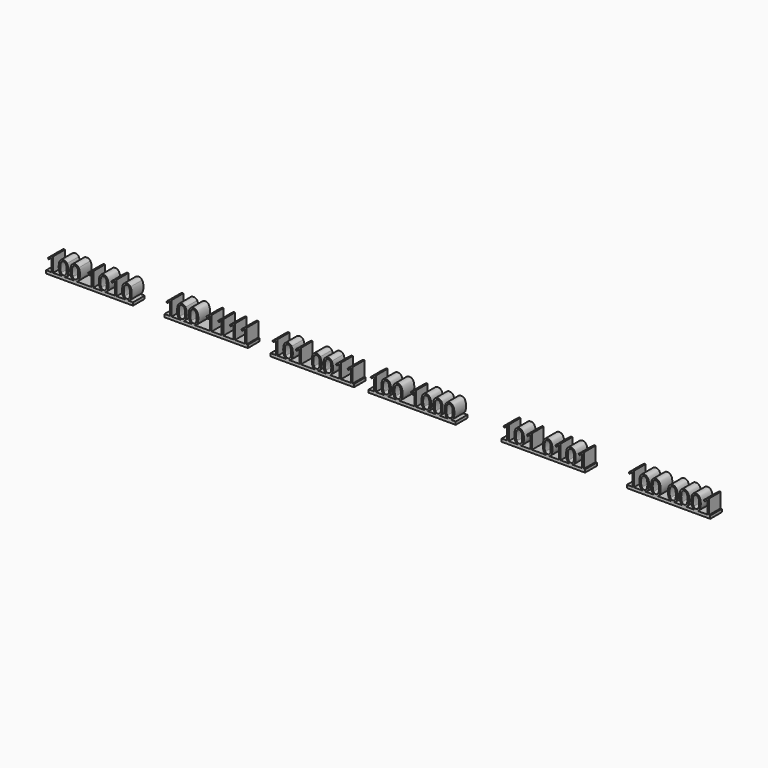
from build123d import *

# Parameters (mm, degrees)
F1_DEPTH       = 25
F2_TEXT_SIZE   = 22.2222222222
F2_TEXT_SIZE_2 = 29.1666666667
F3_DEPTH       = 3


# Not quite as in the source:
# - Text() gives the source's letters only with a copy of the font that has no kerning and outlines rounded to 1/6400 em; it was checked with that copy


with BuildPart() as f1:
    # F0 (on Front) → F1 (new body)
    with BuildSketch(Plane.XZ):
        with BuildLine():
            Line((848.3515024185, 0), (838.9765024185, 0))
            Line((838.9765024185, 0), (838.9765024185, -5))
            Line((838.9765024185, -5), (981.4786725574, -5))
            Line((981.4786725574, -5), (981.4786725574, 0))
            Line((981.4786725574, 0), (979.2271534602, 0))
            Line((979.2271534602, 0), (976.4819277657, 0))
            Line((976.4819277657, 0), (959.6650058477, 0))
            add(Edge.make_bspline(
                [(959.6650058477, 0), (958.5265612688, -0.341796875), (957.1568409602, -0.341796875)],
                knots=[0.6716946069, 0.6716946069, 0.6716946069, 1, 1, 1], degree=2))
            add(Edge.make_bspline(
                [(957.1568409602, -0.341796875), (955.8595624514, -0.341796875), (954.7635928789, 0)],
                knots=[0, 0, 0, 0.3244428423, 0.3244428423, 0.3244428423], degree=2))
            Line((954.7635928789, 0), (939.8136603616, 0))
            add(Edge.make_bspline(
                [(939.8136603616, 0), (938.6752157827, -0.341796875), (937.3054954741, -0.341796875)],
                knots=[0.6716946069, 0.6716946069, 0.6716946069, 1, 1, 1], degree=2))
            add(Edge.make_bspline(
                [(937.3054954741, -0.341796875), (936.0082169652, -0.341796875), (934.9122473928, 0)],
                knots=[0, 0, 0, 0.3244428423, 0.3244428423, 0.3244428423], degree=2))
            Line((934.9122473928, 0), (919.9623148755, 0))
            add(Edge.make_bspline(
                [(919.9623148755, 0), (918.8238702966, -0.341796875), (917.454149988, -0.341796875)],
                knots=[0.6716946069, 0.6716946069, 0.6716946069, 1, 1, 1], degree=2))
            add(Edge.make_bspline(
                [(917.454149988, -0.341796875), (916.1568714791, -0.341796875), (915.0609019067, 0)],
                knots=[0, 0, 0, 0.3244428423, 0.3244428423, 0.3244428423], degree=2))
            Line((915.0609019067, 0), (891.0886169588, 0))
            add(Edge.make_bspline(
                [(891.0886169588, 0), (889.95017238, -0.341796875), (888.5804520713, -0.341796875)],
                knots=[0.6716946069, 0.6716946069, 0.6716946069, 1, 1, 1], degree=2))
            add(Edge.make_bspline(
                [(888.5804520713, -0.341796875), (887.2831735625, -0.341796875), (886.18720399, 0)],
                knots=[0, 0, 0, 0.3244428423, 0.3244428423, 0.3244428423], degree=2))
            Line((886.18720399, 0), (871.2372714727, 0))
            add(Edge.make_bspline(
                [(871.2372714727, 0), (870.0988268938, -0.341796875), (868.7291065852, -0.341796875)],
                knots=[0.6716946069, 0.6716946069, 0.6716946069, 1, 1, 1], degree=2))
            add(Edge.make_bspline(
                [(868.7291065852, -0.341796875), (867.4318280764, -0.341796875), (866.3358585039, 0)],
                knots=[0, 0, 0, 0.3244428423, 0.3244428423, 0.3244428423], degree=2))
            Line((866.3358585039, 0), (851.096728113, 0))
            Line((851.096728113, 0), (848.3515024185, 0))
        make_face()
        with BuildLine():
            Line((58.6257852614, 0), (49.2507852614, 0))
            Line((49.2507852614, 0), (49.2507852614, -5))
            Line((49.2507852614, -5), (191.7529554003, -5))
            Line((191.7529554003, -5), (191.7529554003, 0))
            Line((191.7529554003, 0), (189.5014363031, 0))
            Line((189.5014363031, 0), (186.7562106086, 0))
            Line((186.7562106086, 0), (169.6500908169, 0))
            Line((169.6500908169, 0), (166.9048651225, 0))
            Line((166.9048651225, 0), (149.7987453308, 0))
            Line((149.7987453308, 0), (147.0535196364, 0))
            Line((147.0535196364, 0), (129.9473998447, 0))
            Line((129.9473998447, 0), (127.2021741503, 0))
            Line((127.2021741503, 0), (101.3628998017, 0))
            add(Edge.make_bspline(
                [(101.3628998017, 0), (100.2244552228, -0.341796875), (98.8547349142, -0.341796875)],
                knots=[0.6716946069, 0.6716946069, 0.6716946069, 1, 1, 1], degree=2))
            add(Edge.make_bspline(
                [(98.8547349142, -0.341796875), (97.5574564053, -0.341796875), (96.4614868329, 0)],
                knots=[0, 0, 0, 0.3244428423, 0.3244428423, 0.3244428423], degree=2))
            Line((96.4614868329, 0), (81.5115543156, 0))
            add(Edge.make_bspline(
                [(81.5115543156, 0), (80.3731097367, -0.341796875), (79.0033894281, -0.341796875)],
                knots=[0.6716946069, 0.6716946069, 0.6716946069, 1, 1, 1], degree=2))
            add(Edge.make_bspline(
                [(79.0033894281, -0.341796875), (77.7061109192, -0.341796875), (76.6101413468, 0)],
                knots=[0, 0, 0, 0.3244428423, 0.3244428423, 0.3244428423], degree=2))
            Line((76.6101413468, 0), (61.3710109558, 0))
            Line((61.3710109558, 0), (58.6257852614, 0))
        make_face()
        with BuildLine():
            add(Edge.make_bspline(
                [(652.6452173127, 0), (650.3631817956, 0.7116918462), (648.9539384842, 2.9052734375)],
                knots=[0.3244428423, 0.3244428423, 0.3244428423, 1, 1, 1], degree=2))
            Line((652.6452173127, 0), (657.5466302815, 0))
            add(Edge.make_bspline(
                [(661.2369245953, 2.8293185764), (659.8758246839, 0.6992974298), (657.5466302815, 0)],
                knots=[0, 0, 0, 0.6716946069, 0.6716946069, 0.6716946069], degree=2))
            add(Edge.make_bspline(
                [(663.2632917828, 12.4294704861), (663.2632917828, 6.0004340278), (661.2369245953, 2.8293185764)],
                knots=[0, 0, 0, 1, 1, 1], degree=2))
            add(Edge.make_bspline(
                [(661.169107755, 21.9048394097), (663.2632917828, 18.6306423611), (663.2632917828, 12.4294704861)],
                knots=[0, 0, 0, 1, 1, 1], degree=2))
            add(Edge.make_bspline(
                [(655.0384653939, 25.1790364583), (659.0749237272, 25.1790364583), (661.169107755, 21.9048394097)],
                knots=[0, 0, 0, 1, 1, 1], degree=2))
            add(Edge.make_bspline(
                [(648.8861216439, 22.0404730903), (650.9043508106, 25.1790364583), (655.0384653939, 25.1790364583)],
                knots=[0, 0, 0, 1, 1, 1], degree=2))
            add(Edge.make_bspline(
                [(646.8678924772, 12.4294704861), (646.8678924772, 18.9019097222), (648.8861216439, 22.0404730903)],
                knots=[0, 0, 0, 1, 1, 1], degree=2))
            add(Edge.make_bspline(
                [(648.9539384842, 2.9052734375), (646.8678924772, 6.15234375), (646.8678924772, 12.4294704861)],
                knots=[0, 0, 0, 1, 1, 1], degree=2))
        make_face()
        with BuildLine():
            add(Edge.make_bspline(
                [(649.7161997689, 12.4294704861), (649.7161997689, 7.0203993056), (650.9884436925, 4.5518663194)],
                knots=[0, 0, 0, 1, 1, 1], degree=2))
            add(Edge.make_bspline(
                [(650.9884436925, 20.2880859375), (649.7161997689, 17.8385416667), (649.7161997689, 12.4294704861)],
                knots=[0, 0, 0, 1, 1, 1], degree=2))
            add(Edge.make_bspline(
                [(655.0384653939, 22.7376302083), (652.2606876161, 22.7376302083), (650.9884436925, 20.2880859375)],
                knots=[0, 0, 0, 1, 1, 1], degree=2))
            add(Edge.make_bspline(
                [(659.1156138314, 20.2528211806), (657.8542206022, 22.7376302083), (655.0384653939, 22.7376302083)],
                knots=[0, 0, 0, 1, 1, 1], degree=2))
            add(Edge.make_bspline(
                [(660.3770070606, 12.4294704861), (660.3770070606, 17.7680121528), (659.1156138314, 20.2528211806)],
                knots=[0, 0, 0, 1, 1, 1], degree=2))
            add(Edge.make_bspline(
                [(659.1156138314, 4.5844184028), (660.3770070606, 7.0855034722), (660.3770070606, 12.4294704861)],
                knots=[0, 0, 0, 1, 1, 1], degree=2))
            add(Edge.make_bspline(
                [(655.0384653939, 2.0833333333), (657.8542206022, 2.0833333333), (659.1156138314, 4.5844184028)],
                knots=[0, 0, 0, 1, 1, 1], degree=2))
            add(Edge.make_bspline(
                [(650.9884436925, 4.5518663194), (652.2606876161, 2.0833333333), (655.0384653939, 2.0833333333)],
                knots=[0, 0, 0, 1, 1, 1], degree=2))
        make_face(mode=Mode.SUBTRACT)
        with BuildLine():
            Line((239.8736006684, 0), (230.4986006684, 0))
            Line((230.4986006684, 0), (230.4986006684, -5))
            Line((230.4986006684, -5), (373.0007708073, -5))
            Line((373.0007708073, -5), (373.0007708073, 0))
            Line((373.0007708073, 0), (370.74925171, 0))
            Line((370.74925171, 0), (368.0040260156, 0))
            Line((368.0040260156, 0), (350.8979062239, 0))
            Line((350.8979062239, 0), (348.1526805295, 0))
            Line((348.1526805295, 0), (331.3357586115, 0))
            add(Edge.make_bspline(
                [(331.3357586115, 0), (330.1973140326, -0.341796875), (328.8275937239, -0.341796875)],
                knots=[0.6716946069, 0.6716946069, 0.6716946069, 1, 1, 1], degree=2))
            add(Edge.make_bspline(
                [(328.8275937239, -0.341796875), (327.5303152151, -0.341796875), (326.4343456427, 0)],
                knots=[0, 0, 0, 0.3244428423, 0.3244428423, 0.3244428423], degree=2))
            Line((326.4343456427, 0), (311.4844131254, 0))
            add(Edge.make_bspline(
                [(311.4844131254, 0), (310.3459685465, -0.341796875), (308.9762482378, -0.341796875)],
                knots=[0.6716946069, 0.6716946069, 0.6716946069, 1, 1, 1], degree=2))
            add(Edge.make_bspline(
                [(308.9762482378, -0.341796875), (307.678969729, -0.341796875), (306.5830001566, 0)],
                knots=[0, 0, 0, 0.3244428423, 0.3244428423, 0.3244428423], degree=2))
            Line((306.5830001566, 0), (282.321517335, 0))
            Line((282.321517335, 0), (279.5762916406, 0))
            Line((279.5762916406, 0), (262.7593697226, 0))
            add(Edge.make_bspline(
                [(262.7593697226, 0), (261.6209251437, -0.341796875), (260.251204835, -0.341796875)],
                knots=[0.6716946069, 0.6716946069, 0.6716946069, 1, 1, 1], degree=2))
            add(Edge.make_bspline(
                [(260.251204835, -0.341796875), (258.9539263262, -0.341796875), (257.8579567538, 0)],
                knots=[0, 0, 0, 0.3244428423, 0.3244428423, 0.3244428423], degree=2))
            Line((257.8579567538, 0), (242.6188263628, 0))
            Line((242.6188263628, 0), (239.8736006684, 0))
        make_face()
        with BuildLine():
            Line((407.5516104698, 0), (398.1766104698, 0))
            Line((398.1766104698, 0), (398.1766104698, -5))
            Line((398.1766104698, -5), (546.6846399837, -5))
            Line((546.6846399837, -5), (546.6846399837, 0))
            Line((546.6846399837, 0), (538.7164593851, 0))
            add(Edge.make_bspline(
                [(538.7164593851, 0), (537.5780148063, -0.341796875), (536.2082944976, -0.341796875)],
                knots=[0.6716946069, 0.6716946069, 0.6716946069, 1, 1, 1], degree=2))
            add(Edge.make_bspline(
                [(536.2082944976, -0.341796875), (534.9110159888, -0.341796875), (533.8150464163, 0)],
                knots=[0, 0, 0, 0.3244428423, 0.3244428423, 0.3244428423], degree=2))
            Line((533.8150464163, 0), (518.865113899, 0))
            add(Edge.make_bspline(
                [(518.865113899, 0), (517.7266693201, -0.341796875), (516.3569490115, -0.341796875)],
                knots=[0.6716946069, 0.6716946069, 0.6716946069, 1, 1, 1], degree=2))
            add(Edge.make_bspline(
                [(516.3569490115, -0.341796875), (515.0596705027, -0.341796875), (513.9637009302, 0)],
                knots=[0, 0, 0, 0.3244428423, 0.3244428423, 0.3244428423], degree=2))
            Line((513.9637009302, 0), (499.0137684129, 0))
            add(Edge.make_bspline(
                [(499.0137684129, 0), (497.875323834, -0.341796875), (496.5056035254, -0.341796875)],
                knots=[0.6716946069, 0.6716946069, 0.6716946069, 1, 1, 1], degree=2))
            add(Edge.make_bspline(
                [(496.5056035254, -0.341796875), (495.2083250165, -0.341796875), (494.1123554441, 0)],
                knots=[0, 0, 0, 0.3244428423, 0.3244428423, 0.3244428423], degree=2))
            Line((494.1123554441, 0), (478.8732250532, 0))
            Line((478.8732250532, 0), (476.1279993587, 0))
            Line((476.1279993587, 0), (450.2887250101, 0))
            add(Edge.make_bspline(
                [(450.2887250101, 0), (449.1502804313, -0.341796875), (447.7805601226, -0.341796875)],
                knots=[0.6716946069, 0.6716946069, 0.6716946069, 1, 1, 1], degree=2))
            add(Edge.make_bspline(
                [(447.7805601226, -0.341796875), (446.4832816138, -0.341796875), (445.3873120413, 0)],
                knots=[0, 0, 0, 0.3244428423, 0.3244428423, 0.3244428423], degree=2))
            Line((445.3873120413, 0), (430.437379524, 0))
            add(Edge.make_bspline(
                [(430.437379524, 0), (429.2989349451, -0.341796875), (427.9292146365, -0.341796875)],
                knots=[0.6716946069, 0.6716946069, 0.6716946069, 1, 1, 1], degree=2))
            add(Edge.make_bspline(
                [(427.9292146365, -0.341796875), (426.6319361277, -0.341796875), (425.5359665552, 0)],
                knots=[0, 0, 0, 0.3244428423, 0.3244428423, 0.3244428423], degree=2))
            Line((425.5359665552, 0), (410.2968361643, 0))
            Line((410.2968361643, 0), (407.5516104698, 0))
        make_face()
        with BuildLine():
            Line((634.6608612272, 0), (625.2858612272, 0))
            Line((625.2858612272, 0), (625.2858612272, -5))
            Line((625.2858612272, -5), (767.7880313661, -5))
            Line((767.7880313661, -5), (767.7880313661, 0))
            Line((767.7880313661, 0), (765.5365122689, 0))
            Line((765.5365122689, 0), (762.7912865745, 0))
            Line((762.7912865745, 0), (745.9743646565, 0))
            add(Edge.make_bspline(
                [(745.9743646565, 0), (744.8359200776, -0.341796875), (743.4661997689, -0.341796875)],
                knots=[0.6716946069, 0.6716946069, 0.6716946069, 1, 1, 1], degree=2))
            add(Edge.make_bspline(
                [(743.4661997689, -0.341796875), (742.1689212601, -0.341796875), (741.0729516877, 0)],
                knots=[0, 0, 0, 0.3244428423, 0.3244428423, 0.3244428423], degree=2))
            Line((741.0729516877, 0), (725.8338212967, 0))
            Line((725.8338212967, 0), (723.0885956022, 0))
            Line((723.0885956022, 0), (706.2716736842, 0))
            add(Edge.make_bspline(
                [(706.2716736842, 0), (705.1332291054, -0.341796875), (703.7635087967, -0.341796875)],
                knots=[0.6716946069, 0.6716946069, 0.6716946069, 1, 1, 1], degree=2))
            add(Edge.make_bspline(
                [(703.7635087967, -0.341796875), (702.4662302879, -0.341796875), (701.3702607154, 0)],
                knots=[0, 0, 0, 0.3244428423, 0.3244428423, 0.3244428423], degree=2))
            Line((701.3702607154, 0), (677.1087778939, 0))
            Line((677.1087778939, 0), (674.3635521995, 0))
            Line((674.3635521995, 0), (657.5466302815, 0))
            add(Edge.make_bspline(
                [(657.5466302815, 0), (656.4081857026, -0.341796875), (655.0384653939, -0.341796875)],
                knots=[0.6716946069, 0.6716946069, 0.6716946069, 1, 1, 1], degree=2))
            add(Edge.make_bspline(
                [(655.0384653939, -0.341796875), (653.7411868851, -0.341796875), (652.6452173127, 0)],
                knots=[0, 0, 0, 0.3244428423, 0.3244428423, 0.3244428423], degree=2))
            Line((652.6452173127, 0), (637.4060869217, 0))
            Line((637.4060869217, 0), (634.6608612272, 0))
        make_face()
        with BuildLine():
            Line((934.9122473928, 0), (939.8136603616, 0))
            add(Edge.make_bspline(
                [(943.5039546755, 2.8293185764), (942.142854764, 0.6992974298), (939.8136603616, 0)],
                knots=[0, 0, 0, 0.6716946069, 0.6716946069, 0.6716946069], degree=2))
            add(Edge.make_bspline(
                [(945.530321863, 12.4294704861), (945.530321863, 6.0004340278), (943.5039546755, 2.8293185764)],
                knots=[0, 0, 0, 1, 1, 1], degree=2))
            add(Edge.make_bspline(
                [(943.4361378352, 21.9048394097), (945.530321863, 18.6306423611), (945.530321863, 12.4294704861)],
                knots=[0, 0, 0, 1, 1, 1], degree=2))
            add(Edge.make_bspline(
                [(937.3054954741, 25.1790364583), (941.3419538074, 25.1790364583), (943.4361378352, 21.9048394097)],
                knots=[0, 0, 0, 1, 1, 1], degree=2))
            add(Edge.make_bspline(
                [(931.1531517241, 22.0404730903), (933.1713808907, 25.1790364583), (937.3054954741, 25.1790364583)],
                knots=[0, 0, 0, 1, 1, 1], degree=2))
            add(Edge.make_bspline(
                [(929.1349225574, 12.4294704861), (929.1349225574, 18.9019097222), (931.1531517241, 22.0404730903)],
                knots=[0, 0, 0, 1, 1, 1], degree=2))
            add(Edge.make_bspline(
                [(931.2209685644, 2.9052734375), (929.1349225574, 6.15234375), (929.1349225574, 12.4294704861)],
                knots=[0, 0, 0, 1, 1, 1], degree=2))
            add(Edge.make_bspline(
                [(934.9122473928, 0), (932.6302118757, 0.7116918462), (931.2209685644, 2.9052734375)],
                knots=[0.3244428423, 0.3244428423, 0.3244428423, 1, 1, 1], degree=2))
        make_face()
        with BuildLine():
            add(Edge.make_bspline(
                [(931.9832298491, 12.4294704861), (931.9832298491, 7.0203993056), (933.2554737727, 4.5518663194)],
                knots=[0, 0, 0, 1, 1, 1], degree=2))
            add(Edge.make_bspline(
                [(933.2554737727, 20.2880859375), (931.9832298491, 17.8385416667), (931.9832298491, 12.4294704861)],
                knots=[0, 0, 0, 1, 1, 1], degree=2))
            add(Edge.make_bspline(
                [(937.3054954741, 22.7376302083), (934.5277176963, 22.7376302083), (933.2554737727, 20.2880859375)],
                knots=[0, 0, 0, 1, 1, 1], degree=2))
            add(Edge.make_bspline(
                [(941.3826439116, 20.2528211806), (940.1212506824, 22.7376302083), (937.3054954741, 22.7376302083)],
                knots=[0, 0, 0, 1, 1, 1], degree=2))
            add(Edge.make_bspline(
                [(942.6440371407, 12.4294704861), (942.6440371407, 17.7680121528), (941.3826439116, 20.2528211806)],
                knots=[0, 0, 0, 1, 1, 1], degree=2))
            add(Edge.make_bspline(
                [(941.3826439116, 4.5844184028), (942.6440371407, 7.0855034722), (942.6440371407, 12.4294704861)],
                knots=[0, 0, 0, 1, 1, 1], degree=2))
            add(Edge.make_bspline(
                [(937.3054954741, 2.0833333333), (940.1212506824, 2.0833333333), (941.3826439116, 4.5844184028)],
                knots=[0, 0, 0, 1, 1, 1], degree=2))
            add(Edge.make_bspline(
                [(933.2554737727, 4.5518663194), (934.5277176963, 2.0833333333), (937.3054954741, 2.0833333333)],
                knots=[0, 0, 0, 1, 1, 1], degree=2))
        make_face(mode=Mode.SUBTRACT)
        with BuildLine():
            Line((723.0885956022, 0), (725.8338212967, 0))
            Line((725.8338212967, 0), (725.8338212967, 24.7884114583))
            Line((725.8338212967, 24.7884114583), (723.4629445606, 24.7884114583))
            Line((723.4629445606, 24.7884114583), (716.9036997689, 19.7157118056))
            Line((716.9036997689, 19.7157118056), (718.395670255, 17.7842881944))
            add(Edge.make_bspline(
                [(722.4294159147, 21.0910373264), (721.9872501161, 20.703125), (718.395670255, 17.7842881944)],
                knots=[0, 0, 0, 1, 1, 1], degree=2))
            add(Edge.make_bspline(
                [(723.2242292828, 21.8370225694), (722.8715817134, 21.4789496528), (722.4294159147, 21.0910373264)],
                knots=[0, 0, 0, 1, 1, 1], degree=2))
            add(Edge.make_bspline(
                [(723.0885956022, 17.6649305556), (723.0885956022, 19.873046875), (723.2242292828, 21.8370225694)],
                knots=[0, 0, 0, 1, 1, 1], degree=2))
            Line((723.0885956022, 17.6649305556), (723.0885956022, 0))
        make_face()
        with BuildLine():
            Line((186.7562106086, 0), (189.5014363031, 0))
            Line((189.5014363031, 0), (189.5014363031, 24.7884114583))
            Line((189.5014363031, 24.7884114583), (187.1305595669, 24.7884114583))
            Line((187.1305595669, 24.7884114583), (180.5713147753, 19.7157118056))
            Line((180.5713147753, 19.7157118056), (182.0632852614, 17.7842881944))
            add(Edge.make_bspline(
                [(186.0970309211, 21.0910373264), (185.6548651225, 20.703125), (182.0632852614, 17.7842881944)],
                knots=[0, 0, 0, 1, 1, 1], degree=2))
            add(Edge.make_bspline(
                [(186.8918442892, 21.8370225694), (186.5391967197, 21.4789496528), (186.0970309211, 21.0910373264)],
                knots=[0, 0, 0, 1, 1, 1], degree=2))
            add(Edge.make_bspline(
                [(186.7562106086, 17.6649305556), (186.7562106086, 19.873046875), (186.8918442892, 21.8370225694)],
                knots=[0, 0, 0, 1, 1, 1], degree=2))
            Line((186.7562106086, 17.6649305556), (186.7562106086, 0))
        make_face()
        with BuildLine():
            add(Edge.make_bspline(
                [(499.0137684129, 0), (497.875323834, -0.341796875), (496.5056035254, -0.341796875)],
                knots=[0.6716946069, 0.6716946069, 0.6716946069, 1, 1, 1], degree=2))
            Line((499.0137684129, 0), (494.1123554441, 0))
            add(Edge.make_bspline(
                [(496.5056035254, -0.341796875), (495.2083250165, -0.341796875), (494.1123554441, 0)],
                knots=[0, 0, 0, 0.3244428423, 0.3244428423, 0.3244428423], degree=2))
        make_face()
        with BuildLine():
            Line((919.9623148755, 0), (915.0609019067, 0))
            add(Edge.make_bspline(
                [(917.454149988, -0.341796875), (916.1568714791, -0.341796875), (915.0609019067, 0)],
                knots=[0, 0, 0, 0.3244428423, 0.3244428423, 0.3244428423], degree=2))
            add(Edge.make_bspline(
                [(919.9623148755, 0), (918.8238702966, -0.341796875), (917.454149988, -0.341796875)],
                knots=[0.6716946069, 0.6716946069, 0.6716946069, 1, 1, 1], degree=2))
        make_face()
        with BuildLine():
            add(Edge.make_bspline(
                [(425.5359665552, 0), (423.2539310381, 0.7116918462), (421.8446877268, 2.9052734375)],
                knots=[0.3244428423, 0.3244428423, 0.3244428423, 1, 1, 1], degree=2))
            Line((425.5359665552, 0), (430.437379524, 0))
            add(Edge.make_bspline(
                [(434.1276738379, 2.8293185764), (432.7665739264, 0.6992974298), (430.437379524, 0)],
                knots=[0, 0, 0, 0.6716946069, 0.6716946069, 0.6716946069], degree=2))
            add(Edge.make_bspline(
                [(436.1540410254, 12.4294704861), (436.1540410254, 6.0004340278), (434.1276738379, 2.8293185764)],
                knots=[0, 0, 0, 1, 1, 1], degree=2))
            add(Edge.make_bspline(
                [(434.0598569976, 21.9048394097), (436.1540410254, 18.6306423611), (436.1540410254, 12.4294704861)],
                knots=[0, 0, 0, 1, 1, 1], degree=2))
            add(Edge.make_bspline(
                [(427.9292146365, 25.1790364583), (431.9656729698, 25.1790364583), (434.0598569976, 21.9048394097)],
                knots=[0, 0, 0, 1, 1, 1], degree=2))
            add(Edge.make_bspline(
                [(421.7768708865, 22.0404730903), (423.7951000532, 25.1790364583), (427.9292146365, 25.1790364583)],
                knots=[0, 0, 0, 1, 1, 1], degree=2))
            add(Edge.make_bspline(
                [(419.7586417198, 12.4294704861), (419.7586417198, 18.9019097222), (421.7768708865, 22.0404730903)],
                knots=[0, 0, 0, 1, 1, 1], degree=2))
            add(Edge.make_bspline(
                [(421.8446877268, 2.9052734375), (419.7586417198, 6.15234375), (419.7586417198, 12.4294704861)],
                knots=[0, 0, 0, 1, 1, 1], degree=2))
        make_face()
        with BuildLine():
            add(Edge.make_bspline(
                [(422.6069490115, 12.4294704861), (422.6069490115, 7.0203993056), (423.8791929351, 4.5518663194)],
                knots=[0, 0, 0, 1, 1, 1], degree=2))
            add(Edge.make_bspline(
                [(423.8791929351, 20.2880859375), (422.6069490115, 17.8385416667), (422.6069490115, 12.4294704861)],
                knots=[0, 0, 0, 1, 1, 1], degree=2))
            add(Edge.make_bspline(
                [(427.9292146365, 22.7376302083), (425.1514368587, 22.7376302083), (423.8791929351, 20.2880859375)],
                knots=[0, 0, 0, 1, 1, 1], degree=2))
            add(Edge.make_bspline(
                [(432.006363074, 20.2528211806), (430.7449698448, 22.7376302083), (427.9292146365, 22.7376302083)],
                knots=[0, 0, 0, 1, 1, 1], degree=2))
            add(Edge.make_bspline(
                [(433.2677563032, 12.4294704861), (433.2677563032, 17.7680121528), (432.006363074, 20.2528211806)],
                knots=[0, 0, 0, 1, 1, 1], degree=2))
            add(Edge.make_bspline(
                [(432.006363074, 4.5844184028), (433.2677563032, 7.0855034722), (433.2677563032, 12.4294704861)],
                knots=[0, 0, 0, 1, 1, 1], degree=2))
            add(Edge.make_bspline(
                [(427.9292146365, 2.0833333333), (430.7449698448, 2.0833333333), (432.006363074, 4.5844184028)],
                knots=[0, 0, 0, 1, 1, 1], degree=2))
            add(Edge.make_bspline(
                [(423.8791929351, 4.5518663194), (425.1514368587, 2.0833333333), (427.9292146365, 2.0833333333)],
                knots=[0, 0, 0, 1, 1, 1], degree=2))
        make_face(mode=Mode.SUBTRACT)
        with BuildLine():
            Line((239.8736006684, 17.6649305556), (239.8736006684, 0))
            Line((239.8736006684, 0), (242.6188263628, 0))
            Line((242.6188263628, 0), (242.6188263628, 24.7884114583))
            Line((242.6188263628, 24.7884114583), (240.2479496267, 24.7884114583))
            Line((240.2479496267, 24.7884114583), (233.688704835, 19.7157118056))
            Line((233.688704835, 19.7157118056), (235.1806753212, 17.7842881944))
            add(Edge.make_bspline(
                [(239.2144209809, 21.0910373264), (238.7722551823, 20.703125), (235.1806753212, 17.7842881944)],
                knots=[0, 0, 0, 1, 1, 1], degree=2))
            add(Edge.make_bspline(
                [(240.0092343489, 21.8370225694), (239.6565867795, 21.4789496528), (239.2144209809, 21.0910373264)],
                knots=[0, 0, 0, 1, 1, 1], degree=2))
            add(Edge.make_bspline(
                [(239.8736006684, 17.6649305556), (239.8736006684, 19.873046875), (240.0092343489, 21.8370225694)],
                knots=[0, 0, 0, 1, 1, 1], degree=2))
        make_face()
        with BuildLine():
            add(Edge.make_bspline(
                [(745.9743646565, 0), (744.8359200776, -0.341796875), (743.4661997689, -0.341796875)],
                knots=[0.6716946069, 0.6716946069, 0.6716946069, 1, 1, 1], degree=2))
            Line((745.9743646565, 0), (741.0729516877, 0))
            add(Edge.make_bspline(
                [(743.4661997689, -0.341796875), (742.1689212601, -0.341796875), (741.0729516877, 0)],
                knots=[0, 0, 0, 0.3244428423, 0.3244428423, 0.3244428423], degree=2))
        make_face()
        with BuildLine():
            Line((513.9637009302, 0), (518.865113899, 0))
            add(Edge.make_bspline(
                [(522.5554082129, 2.8293185764), (521.1943083014, 0.6992974298), (518.865113899, 0)],
                knots=[0, 0, 0, 0.6716946069, 0.6716946069, 0.6716946069], degree=2))
            add(Edge.make_bspline(
                [(524.5817754004, 12.4294704861), (524.5817754004, 6.0004340278), (522.5554082129, 2.8293185764)],
                knots=[0, 0, 0, 1, 1, 1], degree=2))
            add(Edge.make_bspline(
                [(522.4875913726, 21.9048394097), (524.5817754004, 18.6306423611), (524.5817754004, 12.4294704861)],
                knots=[0, 0, 0, 1, 1, 1], degree=2))
            add(Edge.make_bspline(
                [(516.3569490115, 25.1790364583), (520.3934073448, 25.1790364583), (522.4875913726, 21.9048394097)],
                knots=[0, 0, 0, 1, 1, 1], degree=2))
            add(Edge.make_bspline(
                [(510.2046052615, 22.0404730903), (512.2228344282, 25.1790364583), (516.3569490115, 25.1790364583)],
                knots=[0, 0, 0, 1, 1, 1], degree=2))
            add(Edge.make_bspline(
                [(508.1863760948, 12.4294704861), (508.1863760948, 18.9019097222), (510.2046052615, 22.0404730903)],
                knots=[0, 0, 0, 1, 1, 1], degree=2))
            add(Edge.make_bspline(
                [(510.2724221018, 2.9052734375), (508.1863760948, 6.15234375), (508.1863760948, 12.4294704861)],
                knots=[0, 0, 0, 1, 1, 1], degree=2))
            add(Edge.make_bspline(
                [(513.9637009302, 0), (511.6816654131, 0.7116918462), (510.2724221018, 2.9052734375)],
                knots=[0.3244428423, 0.3244428423, 0.3244428423, 1, 1, 1], degree=2))
        make_face()
        with BuildLine():
            add(Edge.make_bspline(
                [(511.0346833865, 12.4294704861), (511.0346833865, 7.0203993056), (512.3069273101, 4.5518663194)],
                knots=[0, 0, 0, 1, 1, 1], degree=2))
            add(Edge.make_bspline(
                [(512.3069273101, 20.2880859375), (511.0346833865, 17.8385416667), (511.0346833865, 12.4294704861)],
                knots=[0, 0, 0, 1, 1, 1], degree=2))
            add(Edge.make_bspline(
                [(516.3569490115, 22.7376302083), (513.5791712337, 22.7376302083), (512.3069273101, 20.2880859375)],
                knots=[0, 0, 0, 1, 1, 1], degree=2))
            add(Edge.make_bspline(
                [(520.434097449, 20.2528211806), (519.1727042198, 22.7376302083), (516.3569490115, 22.7376302083)],
                knots=[0, 0, 0, 1, 1, 1], degree=2))
            add(Edge.make_bspline(
                [(521.6954906782, 12.4294704861), (521.6954906782, 17.7680121528), (520.434097449, 20.2528211806)],
                knots=[0, 0, 0, 1, 1, 1], degree=2))
            add(Edge.make_bspline(
                [(520.434097449, 4.5844184028), (521.6954906782, 7.0855034722), (521.6954906782, 12.4294704861)],
                knots=[0, 0, 0, 1, 1, 1], degree=2))
            add(Edge.make_bspline(
                [(516.3569490115, 2.0833333333), (519.1727042198, 2.0833333333), (520.434097449, 4.5844184028)],
                knots=[0, 0, 0, 1, 1, 1], degree=2))
            add(Edge.make_bspline(
                [(512.3069273101, 4.5518663194), (513.5791712337, 2.0833333333), (516.3569490115, 2.0833333333)],
                knots=[0, 0, 0, 1, 1, 1], degree=2))
        make_face(mode=Mode.SUBTRACT)
        with BuildLine():
            add(Edge.make_bspline(
                [(76.6101413468, 0), (74.3281058297, 0.7116918462), (72.9188625183, 2.9052734375)],
                knots=[0.3244428423, 0.3244428423, 0.3244428423, 1, 1, 1], degree=2))
            Line((76.6101413468, 0), (81.5115543156, 0))
            add(Edge.make_bspline(
                [(85.2018486294, 2.8293185764), (83.840748718, 0.6992974298), (81.5115543156, 0)],
                knots=[0, 0, 0, 0.6716946069, 0.6716946069, 0.6716946069], degree=2))
            add(Edge.make_bspline(
                [(87.2282158169, 12.4294704861), (87.2282158169, 6.0004340278), (85.2018486294, 2.8293185764)],
                knots=[0, 0, 0, 1, 1, 1], degree=2))
            add(Edge.make_bspline(
                [(85.1340317892, 21.9048394097), (87.2282158169, 18.6306423611), (87.2282158169, 12.4294704861)],
                knots=[0, 0, 0, 1, 1, 1], degree=2))
            add(Edge.make_bspline(
                [(79.0033894281, 25.1790364583), (83.0398477614, 25.1790364583), (85.1340317892, 21.9048394097)],
                knots=[0, 0, 0, 1, 1, 1], degree=2))
            add(Edge.make_bspline(
                [(72.8510456781, 22.0404730903), (74.8692748447, 25.1790364583), (79.0033894281, 25.1790364583)],
                knots=[0, 0, 0, 1, 1, 1], degree=2))
            add(Edge.make_bspline(
                [(70.8328165114, 12.4294704861), (70.8328165114, 18.9019097222), (72.8510456781, 22.0404730903)],
                knots=[0, 0, 0, 1, 1, 1], degree=2))
            add(Edge.make_bspline(
                [(72.9188625183, 2.9052734375), (70.8328165114, 6.15234375), (70.8328165114, 12.4294704861)],
                knots=[0, 0, 0, 1, 1, 1], degree=2))
        make_face()
        with BuildLine():
            add(Edge.make_bspline(
                [(73.6811238031, 12.4294704861), (73.6811238031, 7.0203993056), (74.9533677267, 4.5518663194)],
                knots=[0, 0, 0, 1, 1, 1], degree=2))
            add(Edge.make_bspline(
                [(74.9533677267, 20.2880859375), (73.6811238031, 17.8385416667), (73.6811238031, 12.4294704861)],
                knots=[0, 0, 0, 1, 1, 1], degree=2))
            add(Edge.make_bspline(
                [(79.0033894281, 22.7376302083), (76.2256116503, 22.7376302083), (74.9533677267, 20.2880859375)],
                knots=[0, 0, 0, 1, 1, 1], degree=2))
            add(Edge.make_bspline(
                [(83.0805378656, 20.2528211806), (81.8191446364, 22.7376302083), (79.0033894281, 22.7376302083)],
                knots=[0, 0, 0, 1, 1, 1], degree=2))
            add(Edge.make_bspline(
                [(84.3419310947, 12.4294704861), (84.3419310947, 17.7680121528), (83.0805378656, 20.2528211806)],
                knots=[0, 0, 0, 1, 1, 1], degree=2))
            add(Edge.make_bspline(
                [(83.0805378656, 4.5844184028), (84.3419310947, 7.0855034722), (84.3419310947, 12.4294704861)],
                knots=[0, 0, 0, 1, 1, 1], degree=2))
            add(Edge.make_bspline(
                [(79.0033894281, 2.0833333333), (81.8191446364, 2.0833333333), (83.0805378656, 4.5844184028)],
                knots=[0, 0, 0, 1, 1, 1], degree=2))
            add(Edge.make_bspline(
                [(74.9533677267, 4.5518663194), (76.2256116503, 2.0833333333), (79.0033894281, 2.0833333333)],
                knots=[0, 0, 0, 1, 1, 1], degree=2))
        make_face(mode=Mode.SUBTRACT)
        with BuildLine():
            Line((533.8150464163, 0), (538.7164593851, 0))
            add(Edge.make_bspline(
                [(542.406753699, 2.8293185764), (541.0456537875, 0.6992974298), (538.7164593851, 0)],
                knots=[0, 0, 0, 0.6716946069, 0.6716946069, 0.6716946069], degree=2))
            add(Edge.make_bspline(
                [(544.4331208865, 12.4294704861), (544.4331208865, 6.0004340278), (542.406753699, 2.8293185764)],
                knots=[0, 0, 0, 1, 1, 1], degree=2))
            add(Edge.make_bspline(
                [(542.3389368587, 21.9048394097), (544.4331208865, 18.6306423611), (544.4331208865, 12.4294704861)],
                knots=[0, 0, 0, 1, 1, 1], degree=2))
            add(Edge.make_bspline(
                [(536.2082944976, 25.1790364583), (540.2447528309, 25.1790364583), (542.3389368587, 21.9048394097)],
                knots=[0, 0, 0, 1, 1, 1], degree=2))
            add(Edge.make_bspline(
                [(530.0559507476, 22.0404730903), (532.0741799143, 25.1790364583), (536.2082944976, 25.1790364583)],
                knots=[0, 0, 0, 1, 1, 1], degree=2))
            add(Edge.make_bspline(
                [(528.0377215809, 12.4294704861), (528.0377215809, 18.9019097222), (530.0559507476, 22.0404730903)],
                knots=[0, 0, 0, 1, 1, 1], degree=2))
            add(Edge.make_bspline(
                [(530.1237675879, 2.9052734375), (528.0377215809, 6.15234375), (528.0377215809, 12.4294704861)],
                knots=[0, 0, 0, 1, 1, 1], degree=2))
            add(Edge.make_bspline(
                [(533.8150464163, 0), (531.5330108992, 0.7116918462), (530.1237675879, 2.9052734375)],
                knots=[0.3244428423, 0.3244428423, 0.3244428423, 1, 1, 1], degree=2))
        make_face()
        with BuildLine():
            add(Edge.make_bspline(
                [(530.8860288726, 12.4294704861), (530.8860288726, 7.0203993056), (532.1582727962, 4.5518663194)],
                knots=[0, 0, 0, 1, 1, 1], degree=2))
            add(Edge.make_bspline(
                [(532.1582727962, 20.2880859375), (530.8860288726, 17.8385416667), (530.8860288726, 12.4294704861)],
                knots=[0, 0, 0, 1, 1, 1], degree=2))
            add(Edge.make_bspline(
                [(536.2082944976, 22.7376302083), (533.4305167198, 22.7376302083), (532.1582727962, 20.2880859375)],
                knots=[0, 0, 0, 1, 1, 1], degree=2))
            add(Edge.make_bspline(
                [(540.2854429351, 20.2528211806), (539.0240497059, 22.7376302083), (536.2082944976, 22.7376302083)],
                knots=[0, 0, 0, 1, 1, 1], degree=2))
            add(Edge.make_bspline(
                [(541.5468361643, 12.4294704861), (541.5468361643, 17.7680121528), (540.2854429351, 20.2528211806)],
                knots=[0, 0, 0, 1, 1, 1], degree=2))
            add(Edge.make_bspline(
                [(540.2854429351, 4.5844184028), (541.5468361643, 7.0855034722), (541.5468361643, 12.4294704861)],
                knots=[0, 0, 0, 1, 1, 1], degree=2))
            add(Edge.make_bspline(
                [(536.2082944976, 2.0833333333), (539.0240497059, 2.0833333333), (540.2854429351, 4.5844184028)],
                knots=[0, 0, 0, 1, 1, 1], degree=2))
            add(Edge.make_bspline(
                [(532.1582727962, 4.5518663194), (533.4305167198, 2.0833333333), (536.2082944976, 2.0833333333)],
                knots=[0, 0, 0, 1, 1, 1], degree=2))
        make_face(mode=Mode.SUBTRACT)
        with BuildLine():
            Line((-57.0601212129, 0), (-52.1587082442, 0))
            add(Edge.make_bspline(
                [(-48.4684139303, 2.8293185764), (-49.8295138417, 0.6992974298), (-52.1587082442, 0)],
                knots=[0, 0, 0, 0.6716946069, 0.6716946069, 0.6716946069], degree=2))
            add(Edge.make_bspline(
                [(-46.4420467428, 12.4294704861), (-46.4420467428, 6.0004340278), (-48.4684139303, 2.8293185764)],
                knots=[0, 0, 0, 1, 1, 1], degree=2))
            add(Edge.make_bspline(
                [(-48.5362307706, 21.9048394097), (-46.4420467428, 18.6306423611), (-46.4420467428, 12.4294704861)],
                knots=[0, 0, 0, 1, 1, 1], degree=2))
            add(Edge.make_bspline(
                [(-54.6668731317, 25.1790364583), (-50.6304147984, 25.1790364583), (-48.5362307706, 21.9048394097)],
                knots=[0, 0, 0, 1, 1, 1], degree=2))
            add(Edge.make_bspline(
                [(-60.8192168817, 22.0404730903), (-58.800987715, 25.1790364583), (-54.6668731317, 25.1790364583)],
                knots=[0, 0, 0, 1, 1, 1], degree=2))
            add(Edge.make_bspline(
                [(-62.8374460484, 12.4294704861), (-62.8374460484, 18.9019097222), (-60.8192168817, 22.0404730903)],
                knots=[0, 0, 0, 1, 1, 1], degree=2))
            add(Edge.make_bspline(
                [(-60.7514000414, 2.9052734375), (-62.8374460484, 6.15234375), (-62.8374460484, 12.4294704861)],
                knots=[0, 0, 0, 1, 1, 1], degree=2))
            add(Edge.make_bspline(
                [(-57.0601212129, 0), (-59.34215673, 0.7116918462), (-60.7514000414, 2.9052734375)],
                knots=[0.3244428423, 0.3244428423, 0.3244428423, 1, 1, 1], degree=2))
        make_face()
        with BuildLine():
            add(Edge.make_bspline(
                [(-59.9891387567, 12.4294704861), (-59.9891387567, 7.0203993056), (-58.7168948331, 4.5518663194)],
                knots=[0, 0, 0, 1, 1, 1], degree=2))
            add(Edge.make_bspline(
                [(-58.7168948331, 20.2880859375), (-59.9891387567, 17.8385416667), (-59.9891387567, 12.4294704861)],
                knots=[0, 0, 0, 1, 1, 1], degree=2))
            add(Edge.make_bspline(
                [(-54.6668731317, 22.7376302083), (-57.4446509095, 22.7376302083), (-58.7168948331, 20.2880859375)],
                knots=[0, 0, 0, 1, 1, 1], degree=2))
            add(Edge.make_bspline(
                [(-50.5897246942, 20.2528211806), (-51.8511179234, 22.7376302083), (-54.6668731317, 22.7376302083)],
                knots=[0, 0, 0, 1, 1, 1], degree=2))
            add(Edge.make_bspline(
                [(-49.328331465, 12.4294704861), (-49.328331465, 17.7680121528), (-50.5897246942, 20.2528211806)],
                knots=[0, 0, 0, 1, 1, 1], degree=2))
            add(Edge.make_bspline(
                [(-50.5897246942, 4.5844184028), (-49.328331465, 7.0855034722), (-49.328331465, 12.4294704861)],
                knots=[0, 0, 0, 1, 1, 1], degree=2))
            add(Edge.make_bspline(
                [(-54.6668731317, 2.0833333333), (-51.8511179234, 2.0833333333), (-50.5897246942, 4.5844184028)],
                knots=[0, 0, 0, 1, 1, 1], degree=2))
            add(Edge.make_bspline(
                [(-58.7168948331, 4.5518663194), (-57.4446509095, 2.0833333333), (-54.6668731317, 2.0833333333)],
                knots=[0, 0, 0, 1, 1, 1], degree=2))
        make_face(mode=Mode.SUBTRACT)
        with BuildLine():
            Line((871.2372714727, 0), (866.3358585039, 0))
            add(Edge.make_bspline(
                [(868.7291065852, -0.341796875), (867.4318280764, -0.341796875), (866.3358585039, 0)],
                knots=[0, 0, 0, 0.3244428423, 0.3244428423, 0.3244428423], degree=2))
            add(Edge.make_bspline(
                [(871.2372714727, 0), (870.0988268938, -0.341796875), (868.7291065852, -0.341796875)],
                knots=[0.6716946069, 0.6716946069, 0.6716946069, 1, 1, 1], degree=2))
        make_face()
        with BuildLine():
            Line((-17.3574302407, 0), (-12.4560172719, 0))
            add(Edge.make_bspline(
                [(-8.7657229581, 2.8293185764), (-10.1268228695, 0.6992974298), (-12.4560172719, 0)],
                knots=[0, 0, 0, 0.6716946069, 0.6716946069, 0.6716946069], degree=2))
            add(Edge.make_bspline(
                [(-6.7393557706, 12.4294704861), (-6.7393557706, 6.0004340278), (-8.7657229581, 2.8293185764)],
                knots=[0, 0, 0, 1, 1, 1], degree=2))
            add(Edge.make_bspline(
                [(-8.8335397984, 21.9048394097), (-6.7393557706, 18.6306423611), (-6.7393557706, 12.4294704861)],
                knots=[0, 0, 0, 1, 1, 1], degree=2))
            add(Edge.make_bspline(
                [(-14.9641821595, 25.1790364583), (-10.9277238261, 25.1790364583), (-8.8335397984, 21.9048394097)],
                knots=[0, 0, 0, 1, 1, 1], degree=2))
            add(Edge.make_bspline(
                [(-21.1165259095, 22.0404730903), (-19.0982967428, 25.1790364583), (-14.9641821595, 25.1790364583)],
                knots=[0, 0, 0, 1, 1, 1], degree=2))
            add(Edge.make_bspline(
                [(-23.1347550761, 12.4294704861), (-23.1347550761, 18.9019097222), (-21.1165259095, 22.0404730903)],
                knots=[0, 0, 0, 1, 1, 1], degree=2))
            add(Edge.make_bspline(
                [(-21.0487090692, 2.9052734375), (-23.1347550761, 6.15234375), (-23.1347550761, 12.4294704861)],
                knots=[0, 0, 0, 1, 1, 1], degree=2))
            add(Edge.make_bspline(
                [(-17.3574302407, 0), (-19.6394657578, 0.7116918462), (-21.0487090692, 2.9052734375)],
                knots=[0.3244428423, 0.3244428423, 0.3244428423, 1, 1, 1], degree=2))
        make_face()
        with BuildLine():
            add(Edge.make_bspline(
                [(-20.2864477845, 12.4294704861), (-20.2864477845, 7.0203993056), (-19.0142038609, 4.5518663194)],
                knots=[0, 0, 0, 1, 1, 1], degree=2))
            add(Edge.make_bspline(
                [(-19.0142038609, 20.2880859375), (-20.2864477845, 17.8385416667), (-20.2864477845, 12.4294704861)],
                knots=[0, 0, 0, 1, 1, 1], degree=2))
            add(Edge.make_bspline(
                [(-14.9641821595, 22.7376302083), (-17.7419599372, 22.7376302083), (-19.0142038609, 20.2880859375)],
                knots=[0, 0, 0, 1, 1, 1], degree=2))
            add(Edge.make_bspline(
                [(-10.887033722, 20.2528211806), (-12.1484269511, 22.7376302083), (-14.9641821595, 22.7376302083)],
                knots=[0, 0, 0, 1, 1, 1], degree=2))
            add(Edge.make_bspline(
                [(-9.6256404928, 12.4294704861), (-9.6256404928, 17.7680121528), (-10.887033722, 20.2528211806)],
                knots=[0, 0, 0, 1, 1, 1], degree=2))
            add(Edge.make_bspline(
                [(-10.887033722, 4.5844184028), (-9.6256404928, 7.0855034722), (-9.6256404928, 12.4294704861)],
                knots=[0, 0, 0, 1, 1, 1], degree=2))
            add(Edge.make_bspline(
                [(-14.9641821595, 2.0833333333), (-12.1484269511, 2.0833333333), (-10.887033722, 4.5844184028)],
                knots=[0, 0, 0, 1, 1, 1], degree=2))
            add(Edge.make_bspline(
                [(-19.0142038609, 4.5518663194), (-17.7419599372, 2.0833333333), (-14.9641821595, 2.0833333333)],
                knots=[0, 0, 0, 1, 1, 1], degree=2))
        make_face(mode=Mode.SUBTRACT)
        with BuildLine():
            Line((450.2887250101, 0), (445.3873120413, 0))
            add(Edge.make_bspline(
                [(447.7805601226, -0.341796875), (446.4832816138, -0.341796875), (445.3873120413, 0)],
                knots=[0, 0, 0, 0.3244428423, 0.3244428423, 0.3244428423], degree=2))
            add(Edge.make_bspline(
                [(450.2887250101, 0), (449.1502804313, -0.341796875), (447.7805601226, -0.341796875)],
                knots=[0.6716946069, 0.6716946069, 0.6716946069, 1, 1, 1], degree=2))
        make_face()
        with BuildLine():
            Line((-75.0444772984, 17.6649305556), (-75.0444772984, 0))
            Line((-75.0444772984, 0), (-72.2992516039, 0))
            Line((-72.2992516039, 0), (-72.2992516039, 24.7884114583))
            Line((-72.2992516039, 24.7884114583), (-74.67012834, 24.7884114583))
            Line((-74.67012834, 24.7884114583), (-81.2293731317, 19.7157118056))
            Line((-81.2293731317, 19.7157118056), (-79.7374026456, 17.7842881944))
            add(Edge.make_bspline(
                [(-75.7036569859, 21.0910373264), (-76.1458227845, 20.703125), (-79.7374026456, 17.7842881944)],
                knots=[0, 0, 0, 1, 1, 1], degree=2))
            add(Edge.make_bspline(
                [(-74.9088436178, 21.8370225694), (-75.2614911872, 21.4789496528), (-75.7036569859, 21.0910373264)],
                knots=[0, 0, 0, 1, 1, 1], degree=2))
            add(Edge.make_bspline(
                [(-75.0444772984, 17.6649305556), (-75.0444772984, 19.873046875), (-74.9088436178, 21.8370225694)],
                knots=[0, 0, 0, 1, 1, 1], degree=2))
        make_face()
        with BuildLine():
            Line((891.0886169588, 0), (886.18720399, 0))
            add(Edge.make_bspline(
                [(888.5804520713, -0.341796875), (887.2831735625, -0.341796875), (886.18720399, 0)],
                knots=[0, 0, 0, 0.3244428423, 0.3244428423, 0.3244428423], degree=2))
            add(Edge.make_bspline(
                [(891.0886169588, 0), (889.95017238, -0.341796875), (888.5804520713, -0.341796875)],
                knots=[0.6716946069, 0.6716946069, 0.6716946069, 1, 1, 1], degree=2))
        make_face()
        with BuildLine():
            add(Edge.make_bspline(
                [(445.3873120413, 0), (443.1052765242, 0.7116918462), (441.6960332129, 2.9052734375)],
                knots=[0.3244428423, 0.3244428423, 0.3244428423, 1, 1, 1], degree=2))
            Line((445.3873120413, 0), (450.2887250101, 0))
            add(Edge.make_bspline(
                [(453.979019324, 2.8293185764), (452.6179194125, 0.6992974298), (450.2887250101, 0)],
                knots=[0, 0, 0, 0.6716946069, 0.6716946069, 0.6716946069], degree=2))
            add(Edge.make_bspline(
                [(456.0053865115, 12.4294704861), (456.0053865115, 6.0004340278), (453.979019324, 2.8293185764)],
                knots=[0, 0, 0, 1, 1, 1], degree=2))
            add(Edge.make_bspline(
                [(453.9112024837, 21.9048394097), (456.0053865115, 18.6306423611), (456.0053865115, 12.4294704861)],
                knots=[0, 0, 0, 1, 1, 1], degree=2))
            add(Edge.make_bspline(
                [(447.7805601226, 25.1790364583), (451.8170184559, 25.1790364583), (453.9112024837, 21.9048394097)],
                knots=[0, 0, 0, 1, 1, 1], degree=2))
            add(Edge.make_bspline(
                [(441.6282163726, 22.0404730903), (443.6464455393, 25.1790364583), (447.7805601226, 25.1790364583)],
                knots=[0, 0, 0, 1, 1, 1], degree=2))
            add(Edge.make_bspline(
                [(439.6099872059, 12.4294704861), (439.6099872059, 18.9019097222), (441.6282163726, 22.0404730903)],
                knots=[0, 0, 0, 1, 1, 1], degree=2))
            add(Edge.make_bspline(
                [(441.6960332129, 2.9052734375), (439.6099872059, 6.15234375), (439.6099872059, 12.4294704861)],
                knots=[0, 0, 0, 1, 1, 1], degree=2))
        make_face()
        with BuildLine():
            add(Edge.make_bspline(
                [(442.4582944976, 12.4294704861), (442.4582944976, 7.0203993056), (443.7305384212, 4.5518663194)],
                knots=[0, 0, 0, 1, 1, 1], degree=2))
            add(Edge.make_bspline(
                [(443.7305384212, 20.2880859375), (442.4582944976, 17.8385416667), (442.4582944976, 12.4294704861)],
                knots=[0, 0, 0, 1, 1, 1], degree=2))
            add(Edge.make_bspline(
                [(447.7805601226, 22.7376302083), (445.0027823448, 22.7376302083), (443.7305384212, 20.2880859375)],
                knots=[0, 0, 0, 1, 1, 1], degree=2))
            add(Edge.make_bspline(
                [(451.8577085601, 20.2528211806), (450.5963153309, 22.7376302083), (447.7805601226, 22.7376302083)],
                knots=[0, 0, 0, 1, 1, 1], degree=2))
            add(Edge.make_bspline(
                [(453.1191017893, 12.4294704861), (453.1191017893, 17.7680121528), (451.8577085601, 20.2528211806)],
                knots=[0, 0, 0, 1, 1, 1], degree=2))
            add(Edge.make_bspline(
                [(451.8577085601, 4.5844184028), (453.1191017893, 7.0855034722), (453.1191017893, 12.4294704861)],
                knots=[0, 0, 0, 1, 1, 1], degree=2))
            add(Edge.make_bspline(
                [(447.7805601226, 2.0833333333), (450.5963153309, 2.0833333333), (451.8577085601, 4.5844184028)],
                knots=[0, 0, 0, 1, 1, 1], degree=2))
            add(Edge.make_bspline(
                [(443.7305384212, 4.5518663194), (445.0027823448, 2.0833333333), (447.7805601226, 2.0833333333)],
                knots=[0, 0, 0, 1, 1, 1], degree=2))
        make_face(mode=Mode.SUBTRACT)
        with BuildLine():
            add(Edge.make_bspline(
                [(886.18720399, 0), (883.9051684729, 0.7116918462), (882.4959251616, 2.9052734375)],
                knots=[0.3244428423, 0.3244428423, 0.3244428423, 1, 1, 1], degree=2))
            Line((886.18720399, 0), (891.0886169588, 0))
            add(Edge.make_bspline(
                [(894.7789112727, 2.8293185764), (893.4178113612, 0.6992974298), (891.0886169588, 0)],
                knots=[0, 0, 0, 0.6716946069, 0.6716946069, 0.6716946069], degree=2))
            add(Edge.make_bspline(
                [(896.8052784602, 12.4294704861), (896.8052784602, 6.0004340278), (894.7789112727, 2.8293185764)],
                knots=[0, 0, 0, 1, 1, 1], degree=2))
            add(Edge.make_bspline(
                [(894.7110944324, 21.9048394097), (896.8052784602, 18.6306423611), (896.8052784602, 12.4294704861)],
                knots=[0, 0, 0, 1, 1, 1], degree=2))
            add(Edge.make_bspline(
                [(888.5804520713, 25.1790364583), (892.6169104046, 25.1790364583), (894.7110944324, 21.9048394097)],
                knots=[0, 0, 0, 1, 1, 1], degree=2))
            add(Edge.make_bspline(
                [(882.4281083213, 22.0404730903), (884.446337488, 25.1790364583), (888.5804520713, 25.1790364583)],
                knots=[0, 0, 0, 1, 1, 1], degree=2))
            add(Edge.make_bspline(
                [(880.4098791546, 12.4294704861), (880.4098791546, 18.9019097222), (882.4281083213, 22.0404730903)],
                knots=[0, 0, 0, 1, 1, 1], degree=2))
            add(Edge.make_bspline(
                [(882.4959251616, 2.9052734375), (880.4098791546, 6.15234375), (880.4098791546, 12.4294704861)],
                knots=[0, 0, 0, 1, 1, 1], degree=2))
        make_face()
        with BuildLine():
            add(Edge.make_bspline(
                [(883.2581864463, 12.4294704861), (883.2581864463, 7.0203993056), (884.5304303699, 4.5518663194)],
                knots=[0, 0, 0, 1, 1, 1], degree=2))
            add(Edge.make_bspline(
                [(884.5304303699, 20.2880859375), (883.2581864463, 17.8385416667), (883.2581864463, 12.4294704861)],
                knots=[0, 0, 0, 1, 1, 1], degree=2))
            add(Edge.make_bspline(
                [(888.5804520713, 22.7376302083), (885.8026742935, 22.7376302083), (884.5304303699, 20.2880859375)],
                knots=[0, 0, 0, 1, 1, 1], degree=2))
            add(Edge.make_bspline(
                [(892.6576005088, 20.2528211806), (891.3962072796, 22.7376302083), (888.5804520713, 22.7376302083)],
                knots=[0, 0, 0, 1, 1, 1], degree=2))
            add(Edge.make_bspline(
                [(893.918993738, 12.4294704861), (893.918993738, 17.7680121528), (892.6576005088, 20.2528211806)],
                knots=[0, 0, 0, 1, 1, 1], degree=2))
            add(Edge.make_bspline(
                [(892.6576005088, 4.5844184028), (893.918993738, 7.0855034722), (893.918993738, 12.4294704861)],
                knots=[0, 0, 0, 1, 1, 1], degree=2))
            add(Edge.make_bspline(
                [(888.5804520713, 2.0833333333), (891.3962072796, 2.0833333333), (892.6576005088, 4.5844184028)],
                knots=[0, 0, 0, 1, 1, 1], degree=2))
            add(Edge.make_bspline(
                [(884.5304303699, 4.5518663194), (885.8026742935, 2.0833333333), (888.5804520713, 2.0833333333)],
                knots=[0, 0, 0, 1, 1, 1], degree=2))
        make_face(mode=Mode.SUBTRACT)
        with BuildLine():
            Line((494.1123554441, 0), (499.0137684129, 0))
            add(Edge.make_bspline(
                [(502.7040627268, 2.8293185764), (501.3429628153, 0.6992974298), (499.0137684129, 0)],
                knots=[0, 0, 0, 0.6716946069, 0.6716946069, 0.6716946069], degree=2))
            add(Edge.make_bspline(
                [(504.7304299143, 12.4294704861), (504.7304299143, 6.0004340278), (502.7040627268, 2.8293185764)],
                knots=[0, 0, 0, 1, 1, 1], degree=2))
            add(Edge.make_bspline(
                [(502.6362458865, 21.9048394097), (504.7304299143, 18.6306423611), (504.7304299143, 12.4294704861)],
                knots=[0, 0, 0, 1, 1, 1], degree=2))
            add(Edge.make_bspline(
                [(496.5056035254, 25.1790364583), (500.5420618587, 25.1790364583), (502.6362458865, 21.9048394097)],
                knots=[0, 0, 0, 1, 1, 1], degree=2))
            add(Edge.make_bspline(
                [(490.3532597754, 22.0404730903), (492.371488942, 25.1790364583), (496.5056035254, 25.1790364583)],
                knots=[0, 0, 0, 1, 1, 1], degree=2))
            add(Edge.make_bspline(
                [(488.3350306087, 12.4294704861), (488.3350306087, 18.9019097222), (490.3532597754, 22.0404730903)],
                knots=[0, 0, 0, 1, 1, 1], degree=2))
            add(Edge.make_bspline(
                [(490.4210766157, 2.9052734375), (488.3350306087, 6.15234375), (488.3350306087, 12.4294704861)],
                knots=[0, 0, 0, 1, 1, 1], degree=2))
            add(Edge.make_bspline(
                [(494.1123554441, 0), (491.830319927, 0.7116918462), (490.4210766157, 2.9052734375)],
                knots=[0.3244428423, 0.3244428423, 0.3244428423, 1, 1, 1], degree=2))
        make_face()
        with BuildLine():
            add(Edge.make_bspline(
                [(491.1833379004, 12.4294704861), (491.1833379004, 7.0203993056), (492.455581824, 4.5518663194)],
                knots=[0, 0, 0, 1, 1, 1], degree=2))
            add(Edge.make_bspline(
                [(492.455581824, 20.2880859375), (491.1833379004, 17.8385416667), (491.1833379004, 12.4294704861)],
                knots=[0, 0, 0, 1, 1, 1], degree=2))
            add(Edge.make_bspline(
                [(496.5056035254, 22.7376302083), (493.7278257476, 22.7376302083), (492.455581824, 20.2880859375)],
                knots=[0, 0, 0, 1, 1, 1], degree=2))
            add(Edge.make_bspline(
                [(500.5827519629, 20.2528211806), (499.3213587337, 22.7376302083), (496.5056035254, 22.7376302083)],
                knots=[0, 0, 0, 1, 1, 1], degree=2))
            add(Edge.make_bspline(
                [(501.844145192, 12.4294704861), (501.844145192, 17.7680121528), (500.5827519629, 20.2528211806)],
                knots=[0, 0, 0, 1, 1, 1], degree=2))
            add(Edge.make_bspline(
                [(500.5827519629, 4.5844184028), (501.844145192, 7.0855034722), (501.844145192, 12.4294704861)],
                knots=[0, 0, 0, 1, 1, 1], degree=2))
            add(Edge.make_bspline(
                [(496.5056035254, 2.0833333333), (499.3213587337, 2.0833333333), (500.5827519629, 4.5844184028)],
                knots=[0, 0, 0, 1, 1, 1], degree=2))
            add(Edge.make_bspline(
                [(492.455581824, 4.5518663194), (493.7278257476, 2.0833333333), (496.5056035254, 2.0833333333)],
                knots=[0, 0, 0, 1, 1, 1], degree=2))
        make_face(mode=Mode.SUBTRACT)
        with BuildLine():
            Line((762.7912865745, 0), (765.5365122689, 0))
            Line((765.5365122689, 0), (765.5365122689, 24.7884114583))
            Line((765.5365122689, 24.7884114583), (763.1656355328, 24.7884114583))
            Line((763.1656355328, 24.7884114583), (756.6063907411, 19.7157118056))
            Line((756.6063907411, 19.7157118056), (758.0983612272, 17.7842881944))
            add(Edge.make_bspline(
                [(762.132106887, 21.0910373264), (761.6899410884, 20.703125), (758.0983612272, 17.7842881944)],
                knots=[0, 0, 0, 1, 1, 1], degree=2))
            add(Edge.make_bspline(
                [(762.926920255, 21.8370225694), (762.5742726856, 21.4789496528), (762.132106887, 21.0910373264)],
                knots=[0, 0, 0, 1, 1, 1], degree=2))
            add(Edge.make_bspline(
                [(762.7912865745, 17.6649305556), (762.7912865745, 19.873046875), (762.926920255, 21.8370225694)],
                knots=[0, 0, 0, 1, 1, 1], degree=2))
            Line((762.7912865745, 17.6649305556), (762.7912865745, 0))
        make_face()
        with BuildLine():
            Line((430.437379524, 0), (425.5359665552, 0))
            add(Edge.make_bspline(
                [(427.9292146365, -0.341796875), (426.6319361277, -0.341796875), (425.5359665552, 0)],
                knots=[0, 0, 0, 0.3244428423, 0.3244428423, 0.3244428423], degree=2))
            add(Edge.make_bspline(
                [(430.437379524, 0), (429.2989349451, -0.341796875), (427.9292146365, -0.341796875)],
                knots=[0.6716946069, 0.6716946069, 0.6716946069, 1, 1, 1], degree=2))
        make_face()
        with BuildLine():
            Line((279.5762916406, 17.6649305556), (279.5762916406, 0))
            Line((279.5762916406, 0), (282.321517335, 0))
            Line((282.321517335, 0), (282.321517335, 24.7884114583))
            Line((282.321517335, 24.7884114583), (279.9506405989, 24.7884114583))
            Line((279.9506405989, 24.7884114583), (273.3913958073, 19.7157118056))
            Line((273.3913958073, 19.7157118056), (274.8833662934, 17.7842881944))
            add(Edge.make_bspline(
                [(278.9171119531, 21.0910373264), (278.4749461545, 20.703125), (274.8833662934, 17.7842881944)],
                knots=[0, 0, 0, 1, 1, 1], degree=2))
            add(Edge.make_bspline(
                [(279.7119253212, 21.8370225694), (279.3592777517, 21.4789496528), (278.9171119531, 21.0910373264)],
                knots=[0, 0, 0, 1, 1, 1], degree=2))
            add(Edge.make_bspline(
                [(279.5762916406, 17.6649305556), (279.5762916406, 19.873046875), (279.7119253212, 21.8370225694)],
                knots=[0, 0, 0, 1, 1, 1], degree=2))
        make_face()
        with BuildLine():
            Line((674.3635521995, 17.6649305556), (674.3635521995, 0))
            Line((674.3635521995, 0), (677.1087778939, 0))
            Line((677.1087778939, 0), (677.1087778939, 24.7884114583))
            Line((677.1087778939, 24.7884114583), (674.7379011578, 24.7884114583))
            Line((674.7379011578, 24.7884114583), (668.1786563661, 19.7157118056))
            Line((668.1786563661, 19.7157118056), (669.6706268522, 17.7842881944))
            add(Edge.make_bspline(
                [(673.704372512, 21.0910373264), (673.2622067134, 20.703125), (669.6706268522, 17.7842881944)],
                knots=[0, 0, 0, 1, 1, 1], degree=2))
            add(Edge.make_bspline(
                [(674.49918588, 21.8370225694), (674.1465383106, 21.4789496528), (673.704372512, 21.0910373264)],
                knots=[0, 0, 0, 1, 1, 1], degree=2))
            add(Edge.make_bspline(
                [(674.3635521995, 17.6649305556), (674.3635521995, 19.873046875), (674.49918588, 21.8370225694)],
                knots=[0, 0, 0, 1, 1, 1], degree=2))
        make_face()
        with BuildLine():
            add(Edge.make_bspline(
                [(915.0609019067, 0), (912.7788663896, 0.7116918462), (911.3696230782, 2.9052734375)],
                knots=[0.3244428423, 0.3244428423, 0.3244428423, 1, 1, 1], degree=2))
            Line((915.0609019067, 0), (919.9623148755, 0))
            add(Edge.make_bspline(
                [(923.6526091894, 2.8293185764), (922.2915092779, 0.6992974298), (919.9623148755, 0)],
                knots=[0, 0, 0, 0.6716946069, 0.6716946069, 0.6716946069], degree=2))
            add(Edge.make_bspline(
                [(925.6789763769, 12.4294704861), (925.6789763769, 6.0004340278), (923.6526091894, 2.8293185764)],
                knots=[0, 0, 0, 1, 1, 1], degree=2))
            add(Edge.make_bspline(
                [(923.5847923491, 21.9048394097), (925.6789763769, 18.6306423611), (925.6789763769, 12.4294704861)],
                knots=[0, 0, 0, 1, 1, 1], degree=2))
            add(Edge.make_bspline(
                [(917.454149988, 25.1790364583), (921.4906083213, 25.1790364583), (923.5847923491, 21.9048394097)],
                knots=[0, 0, 0, 1, 1, 1], degree=2))
            add(Edge.make_bspline(
                [(911.301806238, 22.0404730903), (913.3200354046, 25.1790364583), (917.454149988, 25.1790364583)],
                knots=[0, 0, 0, 1, 1, 1], degree=2))
            add(Edge.make_bspline(
                [(909.2835770713, 12.4294704861), (909.2835770713, 18.9019097222), (911.301806238, 22.0404730903)],
                knots=[0, 0, 0, 1, 1, 1], degree=2))
            add(Edge.make_bspline(
                [(911.3696230782, 2.9052734375), (909.2835770713, 6.15234375), (909.2835770713, 12.4294704861)],
                knots=[0, 0, 0, 1, 1, 1], degree=2))
        make_face()
        with BuildLine():
            add(Edge.make_bspline(
                [(912.131884363, 12.4294704861), (912.131884363, 7.0203993056), (913.4041282866, 4.5518663194)],
                knots=[0, 0, 0, 1, 1, 1], degree=2))
            add(Edge.make_bspline(
                [(913.4041282866, 20.2880859375), (912.131884363, 17.8385416667), (912.131884363, 12.4294704861)],
                knots=[0, 0, 0, 1, 1, 1], degree=2))
            add(Edge.make_bspline(
                [(917.454149988, 22.7376302083), (914.6763722102, 22.7376302083), (913.4041282866, 20.2880859375)],
                knots=[0, 0, 0, 1, 1, 1], degree=2))
            add(Edge.make_bspline(
                [(921.5312984255, 20.2528211806), (920.2699051963, 22.7376302083), (917.454149988, 22.7376302083)],
                knots=[0, 0, 0, 1, 1, 1], degree=2))
            add(Edge.make_bspline(
                [(922.7926916546, 12.4294704861), (922.7926916546, 17.7680121528), (921.5312984255, 20.2528211806)],
                knots=[0, 0, 0, 1, 1, 1], degree=2))
            add(Edge.make_bspline(
                [(921.5312984255, 4.5844184028), (922.7926916546, 7.0855034722), (922.7926916546, 12.4294704861)],
                knots=[0, 0, 0, 1, 1, 1], degree=2))
            add(Edge.make_bspline(
                [(917.454149988, 2.0833333333), (920.2699051963, 2.0833333333), (921.5312984255, 4.5844184028)],
                knots=[0, 0, 0, 1, 1, 1], degree=2))
            add(Edge.make_bspline(
                [(913.4041282866, 4.5518663194), (914.6763722102, 2.0833333333), (917.454149988, 2.0833333333)],
                knots=[0, 0, 0, 1, 1, 1], degree=2))
        make_face(mode=Mode.SUBTRACT)
        with BuildLine():
            Line((81.5115543156, 0), (76.6101413468, 0))
            add(Edge.make_bspline(
                [(79.0033894281, -0.341796875), (77.7061109192, -0.341796875), (76.6101413468, 0)],
                knots=[0, 0, 0, 0.3244428423, 0.3244428423, 0.3244428423], degree=2))
            add(Edge.make_bspline(
                [(81.5115543156, 0), (80.3731097367, -0.341796875), (79.0033894281, -0.341796875)],
                knots=[0.6716946069, 0.6716946069, 0.6716946069, 1, 1, 1], degree=2))
        make_face()
        with BuildLine():
            Line((848.3515024185, 17.6649305556), (848.3515024185, 0))
            Line((848.3515024185, 0), (851.096728113, 0))
            Line((851.096728113, 0), (851.096728113, 24.7884114583))
            Line((851.096728113, 24.7884114583), (848.7258513769, 24.7884114583))
            Line((848.7258513769, 24.7884114583), (842.1666065852, 19.7157118056))
            Line((842.1666065852, 19.7157118056), (843.6585770713, 17.7842881944))
            add(Edge.make_bspline(
                [(847.692322731, 21.0910373264), (847.2501569324, 20.703125), (843.6585770713, 17.7842881944)],
                knots=[0, 0, 0, 1, 1, 1], degree=2))
            add(Edge.make_bspline(
                [(848.4871360991, 21.8370225694), (848.1344885296, 21.4789496528), (847.692322731, 21.0910373264)],
                knots=[0, 0, 0, 1, 1, 1], degree=2))
            add(Edge.make_bspline(
                [(848.3515024185, 17.6649305556), (848.3515024185, 19.873046875), (848.4871360991, 21.8370225694)],
                knots=[0, 0, 0, 1, 1, 1], degree=2))
        make_face()
        with BuildLine():
            add(Edge.make_bspline(
                [(518.865113899, 0), (517.7266693201, -0.341796875), (516.3569490115, -0.341796875)],
                knots=[0.6716946069, 0.6716946069, 0.6716946069, 1, 1, 1], degree=2))
            Line((518.865113899, 0), (513.9637009302, 0))
            add(Edge.make_bspline(
                [(516.3569490115, -0.341796875), (515.0596705027, -0.341796875), (513.9637009302, 0)],
                knots=[0, 0, 0, 0.3244428423, 0.3244428423, 0.3244428423], degree=2))
        make_face()
        with BuildLine():
            Line((348.1526805295, 0), (350.8979062239, 0))
            Line((350.8979062239, 0), (350.8979062239, 24.7884114583))
            Line((350.8979062239, 24.7884114583), (348.5270294878, 24.7884114583))
            Line((348.5270294878, 24.7884114583), (341.9677846962, 19.7157118056))
            Line((341.9677846962, 19.7157118056), (343.4597551823, 17.7842881944))
            add(Edge.make_bspline(
                [(347.493500842, 21.0910373264), (347.0513350434, 20.703125), (343.4597551823, 17.7842881944)],
                knots=[0, 0, 0, 1, 1, 1], degree=2))
            add(Edge.make_bspline(
                [(348.28831421, 21.8370225694), (347.9356666406, 21.4789496528), (347.493500842, 21.0910373264)],
                knots=[0, 0, 0, 1, 1, 1], degree=2))
            add(Edge.make_bspline(
                [(348.1526805295, 17.6649305556), (348.1526805295, 19.873046875), (348.28831421, 21.8370225694)],
                knots=[0, 0, 0, 1, 1, 1], degree=2))
            Line((348.1526805295, 17.6649305556), (348.1526805295, 0))
        make_face()
        with BuildLine():
            add(Edge.make_bspline(
                [(939.8136603616, 0), (938.6752157827, -0.341796875), (937.3054954741, -0.341796875)],
                knots=[0.6716946069, 0.6716946069, 0.6716946069, 1, 1, 1], degree=2))
            Line((939.8136603616, 0), (934.9122473928, 0))
            add(Edge.make_bspline(
                [(937.3054954741, -0.341796875), (936.0082169652, -0.341796875), (934.9122473928, 0)],
                knots=[0, 0, 0, 0.3244428423, 0.3244428423, 0.3244428423], degree=2))
        make_face()
        with BuildLine():
            Line((147.0535196364, 0), (149.7987453308, 0))
            Line((149.7987453308, 0), (149.7987453308, 24.7884114583))
            Line((149.7987453308, 24.7884114583), (147.4278685947, 24.7884114583))
            Line((147.4278685947, 24.7884114583), (140.8686238031, 19.7157118056))
            Line((140.8686238031, 19.7157118056), (142.3605942892, 17.7842881944))
            add(Edge.make_bspline(
                [(146.3943399489, 21.0910373264), (145.9521741503, 20.703125), (142.3605942892, 17.7842881944)],
                knots=[0, 0, 0, 1, 1, 1], degree=2))
            add(Edge.make_bspline(
                [(147.1891533169, 21.8370225694), (146.8365057475, 21.4789496528), (146.3943399489, 21.0910373264)],
                knots=[0, 0, 0, 1, 1, 1], degree=2))
            add(Edge.make_bspline(
                [(147.0535196364, 17.6649305556), (147.0535196364, 19.873046875), (147.1891533169, 21.8370225694)],
                knots=[0, 0, 0, 1, 1, 1], degree=2))
            Line((147.0535196364, 17.6649305556), (147.0535196364, 0))
        make_face()
        with BuildLine():
            Line((166.9048651225, 0), (169.6500908169, 0))
            Line((169.6500908169, 0), (169.6500908169, 24.7884114583))
            Line((169.6500908169, 24.7884114583), (167.2792140808, 24.7884114583))
            Line((167.2792140808, 24.7884114583), (160.7199692892, 19.7157118056))
            Line((160.7199692892, 19.7157118056), (162.2119397753, 17.7842881944))
            add(Edge.make_bspline(
                [(166.245685435, 21.0910373264), (165.8035196364, 20.703125), (162.2119397753, 17.7842881944)],
                knots=[0, 0, 0, 1, 1, 1], degree=2))
            add(Edge.make_bspline(
                [(167.0404988031, 21.8370225694), (166.6878512336, 21.4789496528), (166.245685435, 21.0910373264)],
                knots=[0, 0, 0, 1, 1, 1], degree=2))
            add(Edge.make_bspline(
                [(166.9048651225, 17.6649305556), (166.9048651225, 19.873046875), (167.0404988031, 21.8370225694)],
                knots=[0, 0, 0, 1, 1, 1], degree=2))
            Line((166.9048651225, 17.6649305556), (166.9048651225, 0))
        make_face()
        with BuildLine():
            Line((-143.6208661872, 0), (-152.9958661872, 0))
            Line((-152.9958661872, 0), (-152.9958661872, -5))
            Line((-152.9958661872, -5), (-4.4878366734, -5))
            Line((-4.4878366734, -5), (-4.4878366734, 0))
            Line((-4.4878366734, 0), (-12.4560172719, 0))
            add(Edge.make_bspline(
                [(-12.4560172719, 0), (-13.5944618508, -0.341796875), (-14.9641821595, -0.341796875)],
                knots=[0.6716946069, 0.6716946069, 0.6716946069, 1, 1, 1], degree=2))
            add(Edge.make_bspline(
                [(-14.9641821595, -0.341796875), (-16.2614606683, -0.341796875), (-17.3574302407, 0)],
                knots=[0, 0, 0, 0.3244428423, 0.3244428423, 0.3244428423], degree=2))
            Line((-17.3574302407, 0), (-32.5965606317, 0))
            Line((-32.5965606317, 0), (-35.3417863261, 0))
            Line((-35.3417863261, 0), (-52.1587082442, 0))
            add(Edge.make_bspline(
                [(-52.1587082442, 0), (-53.297152823, -0.341796875), (-54.6668731317, -0.341796875)],
                knots=[0.6716946069, 0.6716946069, 0.6716946069, 1, 1, 1], degree=2))
            add(Edge.make_bspline(
                [(-54.6668731317, -0.341796875), (-55.9641516405, -0.341796875), (-57.0601212129, 0)],
                knots=[0, 0, 0, 0.3244428423, 0.3244428423, 0.3244428423], degree=2))
            Line((-57.0601212129, 0), (-72.2992516039, 0))
            Line((-72.2992516039, 0), (-75.0444772984, 0))
            Line((-75.0444772984, 0), (-100.8837516469, 0))
            add(Edge.make_bspline(
                [(-100.8837516469, 0), (-102.0221962258, -0.341796875), (-103.3919165345, -0.341796875)],
                knots=[0.6716946069, 0.6716946069, 0.6716946069, 1, 1, 1], degree=2))
            add(Edge.make_bspline(
                [(-103.3919165345, -0.341796875), (-104.6891950433, -0.341796875), (-105.7851646157, 0)],
                knots=[0, 0, 0, 0.3244428423, 0.3244428423, 0.3244428423], degree=2))
            Line((-105.7851646157, 0), (-120.735097133, 0))
            add(Edge.make_bspline(
                [(-120.735097133, 0), (-121.8735417119, -0.341796875), (-123.2432620206, -0.341796875)],
                knots=[0.6716946069, 0.6716946069, 0.6716946069, 1, 1, 1], degree=2))
            add(Edge.make_bspline(
                [(-123.2432620206, -0.341796875), (-124.5405405294, -0.341796875), (-125.6365101018, 0)],
                knots=[0, 0, 0, 0.3244428423, 0.3244428423, 0.3244428423], degree=2))
            Line((-125.6365101018, 0), (-140.8756404928, 0))
            Line((-140.8756404928, 0), (-143.6208661872, 0))
        make_face()
        with BuildLine():
            Line((657.5466302815, 0), (652.6452173127, 0))
            add(Edge.make_bspline(
                [(655.0384653939, -0.341796875), (653.7411868851, -0.341796875), (652.6452173127, 0)],
                knots=[0, 0, 0, 0.3244428423, 0.3244428423, 0.3244428423], degree=2))
            add(Edge.make_bspline(
                [(657.5466302815, 0), (656.4081857026, -0.341796875), (655.0384653939, -0.341796875)],
                knots=[0.6716946069, 0.6716946069, 0.6716946069, 1, 1, 1], degree=2))
        make_face()
        with BuildLine():
            add(Edge.make_bspline(
                [(306.5830001566, 0), (304.3009646395, 0.7116918462), (302.8917213281, 2.9052734375)],
                knots=[0.3244428423, 0.3244428423, 0.3244428423, 1, 1, 1], degree=2))
            Line((306.5830001566, 0), (311.4844131254, 0))
            add(Edge.make_bspline(
                [(315.1747074392, 2.8293185764), (313.8136075278, 0.6992974298), (311.4844131254, 0)],
                knots=[0, 0, 0, 0.6716946069, 0.6716946069, 0.6716946069], degree=2))
            add(Edge.make_bspline(
                [(317.2010746267, 12.4294704861), (317.2010746267, 6.0004340278), (315.1747074392, 2.8293185764)],
                knots=[0, 0, 0, 1, 1, 1], degree=2))
            add(Edge.make_bspline(
                [(315.1068905989, 21.9048394097), (317.2010746267, 18.6306423611), (317.2010746267, 12.4294704861)],
                knots=[0, 0, 0, 1, 1, 1], degree=2))
            add(Edge.make_bspline(
                [(308.9762482378, 25.1790364583), (313.0127065712, 25.1790364583), (315.1068905989, 21.9048394097)],
                knots=[0, 0, 0, 1, 1, 1], degree=2))
            add(Edge.make_bspline(
                [(302.8239044878, 22.0404730903), (304.8421336545, 25.1790364583), (308.9762482378, 25.1790364583)],
                knots=[0, 0, 0, 1, 1, 1], degree=2))
            add(Edge.make_bspline(
                [(300.8056753212, 12.4294704861), (300.8056753212, 18.9019097222), (302.8239044878, 22.0404730903)],
                knots=[0, 0, 0, 1, 1, 1], degree=2))
            add(Edge.make_bspline(
                [(302.8917213281, 2.9052734375), (300.8056753212, 6.15234375), (300.8056753212, 12.4294704861)],
                knots=[0, 0, 0, 1, 1, 1], degree=2))
        make_face()
        with BuildLine():
            add(Edge.make_bspline(
                [(303.6539826128, 12.4294704861), (303.6539826128, 7.0203993056), (304.9262265364, 4.5518663194)],
                knots=[0, 0, 0, 1, 1, 1], degree=2))
            add(Edge.make_bspline(
                [(304.9262265364, 20.2880859375), (303.6539826128, 17.8385416667), (303.6539826128, 12.4294704861)],
                knots=[0, 0, 0, 1, 1, 1], degree=2))
            add(Edge.make_bspline(
                [(308.9762482378, 22.7376302083), (306.19847046, 22.7376302083), (304.9262265364, 20.2880859375)],
                knots=[0, 0, 0, 1, 1, 1], degree=2))
            add(Edge.make_bspline(
                [(313.0533966753, 20.2528211806), (311.7920034462, 22.7376302083), (308.9762482378, 22.7376302083)],
                knots=[0, 0, 0, 1, 1, 1], degree=2))
            add(Edge.make_bspline(
                [(314.3147899045, 12.4294704861), (314.3147899045, 17.7680121528), (313.0533966753, 20.2528211806)],
                knots=[0, 0, 0, 1, 1, 1], degree=2))
            add(Edge.make_bspline(
                [(313.0533966753, 4.5844184028), (314.3147899045, 7.0855034722), (314.3147899045, 12.4294704861)],
                knots=[0, 0, 0, 1, 1, 1], degree=2))
            add(Edge.make_bspline(
                [(308.9762482378, 2.0833333333), (311.7920034462, 2.0833333333), (313.0533966753, 4.5844184028)],
                knots=[0, 0, 0, 1, 1, 1], degree=2))
            add(Edge.make_bspline(
                [(304.9262265364, 4.5518663194), (306.19847046, 2.0833333333), (308.9762482378, 2.0833333333)],
                knots=[0, 0, 0, 1, 1, 1], degree=2))
        make_face(mode=Mode.SUBTRACT)
        with BuildLine():
            Line((368.0040260156, 0), (370.74925171, 0))
            Line((370.74925171, 0), (370.74925171, 24.7884114583))
            Line((370.74925171, 24.7884114583), (368.3783749739, 24.7884114583))
            Line((368.3783749739, 24.7884114583), (361.8191301823, 19.7157118056))
            Line((361.8191301823, 19.7157118056), (363.3111006684, 17.7842881944))
            add(Edge.make_bspline(
                [(367.3448463281, 21.0910373264), (366.9026805295, 20.703125), (363.3111006684, 17.7842881944)],
                knots=[0, 0, 0, 1, 1, 1], degree=2))
            add(Edge.make_bspline(
                [(368.1396596962, 21.8370225694), (367.7870121267, 21.4789496528), (367.3448463281, 21.0910373264)],
                knots=[0, 0, 0, 1, 1, 1], degree=2))
            add(Edge.make_bspline(
                [(368.0040260156, 17.6649305556), (368.0040260156, 19.873046875), (368.1396596962, 21.8370225694)],
                knots=[0, 0, 0, 1, 1, 1], degree=2))
            Line((368.0040260156, 17.6649305556), (368.0040260156, 0))
        make_face()
        with BuildLine():
            Line((954.7635928789, 0), (959.6650058477, 0))
            add(Edge.make_bspline(
                [(963.3553001616, 2.8293185764), (961.9942002501, 0.6992974298), (959.6650058477, 0)],
                knots=[0, 0, 0, 0.6716946069, 0.6716946069, 0.6716946069], degree=2))
            add(Edge.make_bspline(
                [(965.3816673491, 12.4294704861), (965.3816673491, 6.0004340278), (963.3553001616, 2.8293185764)],
                knots=[0, 0, 0, 1, 1, 1], degree=2))
            add(Edge.make_bspline(
                [(963.2874833213, 21.9048394097), (965.3816673491, 18.6306423611), (965.3816673491, 12.4294704861)],
                knots=[0, 0, 0, 1, 1, 1], degree=2))
            add(Edge.make_bspline(
                [(957.1568409602, 25.1790364583), (961.1932992935, 25.1790364583), (963.2874833213, 21.9048394097)],
                knots=[0, 0, 0, 1, 1, 1], degree=2))
            add(Edge.make_bspline(
                [(951.0044972102, 22.0404730903), (953.0227263769, 25.1790364583), (957.1568409602, 25.1790364583)],
                knots=[0, 0, 0, 1, 1, 1], degree=2))
            add(Edge.make_bspline(
                [(948.9862680435, 12.4294704861), (948.9862680435, 18.9019097222), (951.0044972102, 22.0404730903)],
                knots=[0, 0, 0, 1, 1, 1], degree=2))
            add(Edge.make_bspline(
                [(951.0723140505, 2.9052734375), (948.9862680435, 6.15234375), (948.9862680435, 12.4294704861)],
                knots=[0, 0, 0, 1, 1, 1], degree=2))
            add(Edge.make_bspline(
                [(954.7635928789, 0), (952.4815573618, 0.7116918462), (951.0723140505, 2.9052734375)],
                knots=[0.3244428423, 0.3244428423, 0.3244428423, 1, 1, 1], degree=2))
        make_face()
        with BuildLine():
            add(Edge.make_bspline(
                [(951.8345753352, 12.4294704861), (951.8345753352, 7.0203993056), (953.1068192588, 4.5518663194)],
                knots=[0, 0, 0, 1, 1, 1], degree=2))
            add(Edge.make_bspline(
                [(953.1068192588, 20.2880859375), (951.8345753352, 17.8385416667), (951.8345753352, 12.4294704861)],
                knots=[0, 0, 0, 1, 1, 1], degree=2))
            add(Edge.make_bspline(
                [(957.1568409602, 22.7376302083), (954.3790631824, 22.7376302083), (953.1068192588, 20.2880859375)],
                knots=[0, 0, 0, 1, 1, 1], degree=2))
            add(Edge.make_bspline(
                [(961.2339893977, 20.2528211806), (959.9725961685, 22.7376302083), (957.1568409602, 22.7376302083)],
                knots=[0, 0, 0, 1, 1, 1], degree=2))
            add(Edge.make_bspline(
                [(962.4953826269, 12.4294704861), (962.4953826269, 17.7680121528), (961.2339893977, 20.2528211806)],
                knots=[0, 0, 0, 1, 1, 1], degree=2))
            add(Edge.make_bspline(
                [(961.2339893977, 4.5844184028), (962.4953826269, 7.0855034722), (962.4953826269, 12.4294704861)],
                knots=[0, 0, 0, 1, 1, 1], degree=2))
            add(Edge.make_bspline(
                [(957.1568409602, 2.0833333333), (959.9725961685, 2.0833333333), (961.2339893977, 4.5844184028)],
                knots=[0, 0, 0, 1, 1, 1], degree=2))
            add(Edge.make_bspline(
                [(953.1068192588, 4.5518663194), (954.3790631824, 2.0833333333), (957.1568409602, 2.0833333333)],
                knots=[0, 0, 0, 1, 1, 1], degree=2))
        make_face(mode=Mode.SUBTRACT)
        with BuildLine():
            add(Edge.make_bspline(
                [(96.4614868329, 0), (94.1794513158, 0.7116918462), (92.7702080044, 2.9052734375)],
                knots=[0.3244428423, 0.3244428423, 0.3244428423, 1, 1, 1], degree=2))
            Line((96.4614868329, 0), (101.3628998017, 0))
            add(Edge.make_bspline(
                [(105.0531941156, 2.8293185764), (103.6920942041, 0.6992974298), (101.3628998017, 0)],
                knots=[0, 0, 0, 0.6716946069, 0.6716946069, 0.6716946069], degree=2))
            add(Edge.make_bspline(
                [(107.0795613031, 12.4294704861), (107.0795613031, 6.0004340278), (105.0531941156, 2.8293185764)],
                knots=[0, 0, 0, 1, 1, 1], degree=2))
            add(Edge.make_bspline(
                [(104.9853772753, 21.9048394097), (107.0795613031, 18.6306423611), (107.0795613031, 12.4294704861)],
                knots=[0, 0, 0, 1, 1, 1], degree=2))
            add(Edge.make_bspline(
                [(98.8547349142, 25.1790364583), (102.8911932475, 25.1790364583), (104.9853772753, 21.9048394097)],
                knots=[0, 0, 0, 1, 1, 1], degree=2))
            add(Edge.make_bspline(
                [(92.7023911642, 22.0404730903), (94.7206203308, 25.1790364583), (98.8547349142, 25.1790364583)],
                knots=[0, 0, 0, 1, 1, 1], degree=2))
            add(Edge.make_bspline(
                [(90.6841619975, 12.4294704861), (90.6841619975, 18.9019097222), (92.7023911642, 22.0404730903)],
                knots=[0, 0, 0, 1, 1, 1], degree=2))
            add(Edge.make_bspline(
                [(92.7702080044, 2.9052734375), (90.6841619975, 6.15234375), (90.6841619975, 12.4294704861)],
                knots=[0, 0, 0, 1, 1, 1], degree=2))
        make_face()
        with BuildLine():
            add(Edge.make_bspline(
                [(93.5324692892, 12.4294704861), (93.5324692892, 7.0203993056), (94.8047132128, 4.5518663194)],
                knots=[0, 0, 0, 1, 1, 1], degree=2))
            add(Edge.make_bspline(
                [(94.8047132128, 20.2880859375), (93.5324692892, 17.8385416667), (93.5324692892, 12.4294704861)],
                knots=[0, 0, 0, 1, 1, 1], degree=2))
            add(Edge.make_bspline(
                [(98.8547349142, 22.7376302083), (96.0769571364, 22.7376302083), (94.8047132128, 20.2880859375)],
                knots=[0, 0, 0, 1, 1, 1], degree=2))
            add(Edge.make_bspline(
                [(102.9318833517, 20.2528211806), (101.6704901225, 22.7376302083), (98.8547349142, 22.7376302083)],
                knots=[0, 0, 0, 1, 1, 1], degree=2))
            add(Edge.make_bspline(
                [(104.1932765808, 12.4294704861), (104.1932765808, 17.7680121528), (102.9318833517, 20.2528211806)],
                knots=[0, 0, 0, 1, 1, 1], degree=2))
            add(Edge.make_bspline(
                [(102.9318833517, 4.5844184028), (104.1932765808, 7.0855034722), (104.1932765808, 12.4294704861)],
                knots=[0, 0, 0, 1, 1, 1], degree=2))
            add(Edge.make_bspline(
                [(98.8547349142, 2.0833333333), (101.6704901225, 2.0833333333), (102.9318833517, 4.5844184028)],
                knots=[0, 0, 0, 1, 1, 1], degree=2))
            add(Edge.make_bspline(
                [(94.8047132128, 4.5518663194), (96.0769571364, 2.0833333333), (98.8547349142, 2.0833333333)],
                knots=[0, 0, 0, 1, 1, 1], degree=2))
        make_face(mode=Mode.SUBTRACT)
        with BuildLine():
            Line((407.5516104698, 17.6649305556), (407.5516104698, 0))
            Line((407.5516104698, 0), (410.2968361643, 0))
            Line((410.2968361643, 0), (410.2968361643, 24.7884114583))
            Line((410.2968361643, 24.7884114583), (407.9259594282, 24.7884114583))
            Line((407.9259594282, 24.7884114583), (401.3667146365, 19.7157118056))
            Line((401.3667146365, 19.7157118056), (402.8586851226, 17.7842881944))
            add(Edge.make_bspline(
                [(406.8924307823, 21.0910373264), (406.4502649837, 20.703125), (402.8586851226, 17.7842881944)],
                knots=[0, 0, 0, 1, 1, 1], degree=2))
            add(Edge.make_bspline(
                [(407.6872441504, 21.8370225694), (407.3345965809, 21.4789496528), (406.8924307823, 21.0910373264)],
                knots=[0, 0, 0, 1, 1, 1], degree=2))
            add(Edge.make_bspline(
                [(407.5516104698, 17.6649305556), (407.5516104698, 19.873046875), (407.6872441504, 21.8370225694)],
                knots=[0, 0, 0, 1, 1, 1], degree=2))
        make_face()
        with BuildLine():
            add(Edge.make_bspline(
                [(959.6650058477, 0), (958.5265612688, -0.341796875), (957.1568409602, -0.341796875)],
                knots=[0.6716946069, 0.6716946069, 0.6716946069, 1, 1, 1], degree=2))
            Line((959.6650058477, 0), (954.7635928789, 0))
            add(Edge.make_bspline(
                [(957.1568409602, -0.341796875), (955.8595624514, -0.341796875), (954.7635928789, 0)],
                knots=[0, 0, 0, 0.3244428423, 0.3244428423, 0.3244428423], degree=2))
        make_face()
        with BuildLine():
            add(Edge.make_bspline(
                [(538.7164593851, 0), (537.5780148063, -0.341796875), (536.2082944976, -0.341796875)],
                knots=[0.6716946069, 0.6716946069, 0.6716946069, 1, 1, 1], degree=2))
            Line((538.7164593851, 0), (533.8150464163, 0))
            add(Edge.make_bspline(
                [(536.2082944976, -0.341796875), (534.9110159888, -0.341796875), (533.8150464163, 0)],
                knots=[0, 0, 0, 0.3244428423, 0.3244428423, 0.3244428423], degree=2))
        make_face()
        with BuildLine():
            Line((101.3628998017, 0), (96.4614868329, 0))
            add(Edge.make_bspline(
                [(98.8547349142, -0.341796875), (97.5574564053, -0.341796875), (96.4614868329, 0)],
                knots=[0, 0, 0, 0.3244428423, 0.3244428423, 0.3244428423], degree=2))
            add(Edge.make_bspline(
                [(101.3628998017, 0), (100.2244552228, -0.341796875), (98.8547349142, -0.341796875)],
                knots=[0.6716946069, 0.6716946069, 0.6716946069, 1, 1, 1], degree=2))
        make_face()
        with BuildLine():
            add(Edge.make_bspline(
                [(257.8579567538, 0), (255.5759212367, 0.7116918462), (254.1666779253, 2.9052734375)],
                knots=[0.3244428423, 0.3244428423, 0.3244428423, 1, 1, 1], degree=2))
            Line((257.8579567538, 0), (262.7593697226, 0))
            add(Edge.make_bspline(
                [(266.4496640364, 2.8293185764), (265.088564125, 0.6992974298), (262.7593697226, 0)],
                knots=[0, 0, 0, 0.6716946069, 0.6716946069, 0.6716946069], degree=2))
            add(Edge.make_bspline(
                [(268.4760312239, 12.4294704861), (268.4760312239, 6.0004340278), (266.4496640364, 2.8293185764)],
                knots=[0, 0, 0, 1, 1, 1], degree=2))
            add(Edge.make_bspline(
                [(266.3818471962, 21.9048394097), (268.4760312239, 18.6306423611), (268.4760312239, 12.4294704861)],
                knots=[0, 0, 0, 1, 1, 1], degree=2))
            add(Edge.make_bspline(
                [(260.251204835, 25.1790364583), (264.2876631684, 25.1790364583), (266.3818471962, 21.9048394097)],
                knots=[0, 0, 0, 1, 1, 1], degree=2))
            add(Edge.make_bspline(
                [(254.098861085, 22.0404730903), (256.1170902517, 25.1790364583), (260.251204835, 25.1790364583)],
                knots=[0, 0, 0, 1, 1, 1], degree=2))
            add(Edge.make_bspline(
                [(252.0806319184, 12.4294704861), (252.0806319184, 18.9019097222), (254.098861085, 22.0404730903)],
                knots=[0, 0, 0, 1, 1, 1], degree=2))
            add(Edge.make_bspline(
                [(254.1666779253, 2.9052734375), (252.0806319184, 6.15234375), (252.0806319184, 12.4294704861)],
                knots=[0, 0, 0, 1, 1, 1], degree=2))
        make_face()
        with BuildLine():
            add(Edge.make_bspline(
                [(254.92893921, 12.4294704861), (254.92893921, 7.0203993056), (256.2011831337, 4.5518663194)],
                knots=[0, 0, 0, 1, 1, 1], degree=2))
            add(Edge.make_bspline(
                [(256.2011831337, 20.2880859375), (254.92893921, 17.8385416667), (254.92893921, 12.4294704861)],
                knots=[0, 0, 0, 1, 1, 1], degree=2))
            add(Edge.make_bspline(
                [(260.251204835, 22.7376302083), (257.4734270573, 22.7376302083), (256.2011831337, 20.2880859375)],
                knots=[0, 0, 0, 1, 1, 1], degree=2))
            add(Edge.make_bspline(
                [(264.3283532725, 20.2528211806), (263.0669600434, 22.7376302083), (260.251204835, 22.7376302083)],
                knots=[0, 0, 0, 1, 1, 1], degree=2))
            add(Edge.make_bspline(
                [(265.5897465017, 12.4294704861), (265.5897465017, 17.7680121528), (264.3283532725, 20.2528211806)],
                knots=[0, 0, 0, 1, 1, 1], degree=2))
            add(Edge.make_bspline(
                [(264.3283532725, 4.5844184028), (265.5897465017, 7.0855034722), (265.5897465017, 12.4294704861)],
                knots=[0, 0, 0, 1, 1, 1], degree=2))
            add(Edge.make_bspline(
                [(260.251204835, 2.0833333333), (263.0669600434, 2.0833333333), (264.3283532725, 4.5844184028)],
                knots=[0, 0, 0, 1, 1, 1], degree=2))
            add(Edge.make_bspline(
                [(256.2011831337, 4.5518663194), (257.4734270573, 2.0833333333), (260.251204835, 2.0833333333)],
                knots=[0, 0, 0, 1, 1, 1], degree=2))
        make_face(mode=Mode.SUBTRACT)
        with BuildLine():
            Line((-35.3417863261, 0), (-32.5965606317, 0))
            Line((-32.5965606317, 0), (-32.5965606317, 24.7884114583))
            Line((-32.5965606317, 24.7884114583), (-34.9674373678, 24.7884114583))
            Line((-34.9674373678, 24.7884114583), (-41.5266821595, 19.7157118056))
            Line((-41.5266821595, 19.7157118056), (-40.0347116734, 17.7842881944))
            add(Edge.make_bspline(
                [(-36.0009660136, 21.0910373264), (-36.4431318122, 20.703125), (-40.0347116734, 17.7842881944)],
                knots=[0, 0, 0, 1, 1, 1], degree=2))
            add(Edge.make_bspline(
                [(-35.2061526456, 21.8370225694), (-35.558800215, 21.4789496528), (-36.0009660136, 21.0910373264)],
                knots=[0, 0, 0, 1, 1, 1], degree=2))
            add(Edge.make_bspline(
                [(-35.3417863261, 17.6649305556), (-35.3417863261, 19.873046875), (-35.2061526456, 21.8370225694)],
                knots=[0, 0, 0, 1, 1, 1], degree=2))
            Line((-35.3417863261, 17.6649305556), (-35.3417863261, 0))
        make_face()
        with BuildLine():
            Line((262.7593697226, 0), (257.8579567538, 0))
            add(Edge.make_bspline(
                [(260.251204835, -0.341796875), (258.9539263262, -0.341796875), (257.8579567538, 0)],
                knots=[0, 0, 0, 0.3244428423, 0.3244428423, 0.3244428423], degree=2))
            add(Edge.make_bspline(
                [(262.7593697226, 0), (261.6209251437, -0.341796875), (260.251204835, -0.341796875)],
                knots=[0.6716946069, 0.6716946069, 0.6716946069, 1, 1, 1], degree=2))
        make_face()
        with BuildLine():
            Line((476.1279993587, 17.6649305556), (476.1279993587, 0))
            Line((476.1279993587, 0), (478.8732250532, 0))
            Line((478.8732250532, 0), (478.8732250532, 24.7884114583))
            Line((478.8732250532, 24.7884114583), (476.502348317, 24.7884114583))
            Line((476.502348317, 24.7884114583), (469.9431035254, 19.7157118056))
            Line((469.9431035254, 19.7157118056), (471.4350740115, 17.7842881944))
            add(Edge.make_bspline(
                [(475.4688196712, 21.0910373264), (475.0266538726, 20.703125), (471.4350740115, 17.7842881944)],
                knots=[0, 0, 0, 1, 1, 1], degree=2))
            add(Edge.make_bspline(
                [(476.2636330393, 21.8370225694), (475.9109854698, 21.4789496528), (475.4688196712, 21.0910373264)],
                knots=[0, 0, 0, 1, 1, 1], degree=2))
            add(Edge.make_bspline(
                [(476.1279993587, 17.6649305556), (476.1279993587, 19.873046875), (476.2636330393, 21.8370225694)],
                knots=[0, 0, 0, 1, 1, 1], degree=2))
        make_face()
        with BuildLine():
            add(Edge.make_bspline(
                [(701.3702607154, 0), (699.0882251983, 0.7116918462), (697.678981887, 2.9052734375)],
                knots=[0.3244428423, 0.3244428423, 0.3244428423, 1, 1, 1], degree=2))
            Line((701.3702607154, 0), (706.2716736842, 0))
            add(Edge.make_bspline(
                [(709.9619679981, 2.8293185764), (708.6008680866, 0.6992974298), (706.2716736842, 0)],
                knots=[0, 0, 0, 0.6716946069, 0.6716946069, 0.6716946069], degree=2))
            add(Edge.make_bspline(
                [(711.9883351856, 12.4294704861), (711.9883351856, 6.0004340278), (709.9619679981, 2.8293185764)],
                knots=[0, 0, 0, 1, 1, 1], degree=2))
            add(Edge.make_bspline(
                [(709.8941511578, 21.9048394097), (711.9883351856, 18.6306423611), (711.9883351856, 12.4294704861)],
                knots=[0, 0, 0, 1, 1, 1], degree=2))
            add(Edge.make_bspline(
                [(703.7635087967, 25.1790364583), (707.79996713, 25.1790364583), (709.8941511578, 21.9048394097)],
                knots=[0, 0, 0, 1, 1, 1], degree=2))
            add(Edge.make_bspline(
                [(697.6111650467, 22.0404730903), (699.6293942134, 25.1790364583), (703.7635087967, 25.1790364583)],
                knots=[0, 0, 0, 1, 1, 1], degree=2))
            add(Edge.make_bspline(
                [(695.59293588, 12.4294704861), (695.59293588, 18.9019097222), (697.6111650467, 22.0404730903)],
                knots=[0, 0, 0, 1, 1, 1], degree=2))
            add(Edge.make_bspline(
                [(697.678981887, 2.9052734375), (695.59293588, 6.15234375), (695.59293588, 12.4294704861)],
                knots=[0, 0, 0, 1, 1, 1], degree=2))
        make_face()
        with BuildLine():
            add(Edge.make_bspline(
                [(698.4412431717, 12.4294704861), (698.4412431717, 7.0203993056), (699.7134870953, 4.5518663194)],
                knots=[0, 0, 0, 1, 1, 1], degree=2))
            add(Edge.make_bspline(
                [(699.7134870953, 20.2880859375), (698.4412431717, 17.8385416667), (698.4412431717, 12.4294704861)],
                knots=[0, 0, 0, 1, 1, 1], degree=2))
            add(Edge.make_bspline(
                [(703.7635087967, 22.7376302083), (700.9857310189, 22.7376302083), (699.7134870953, 20.2880859375)],
                knots=[0, 0, 0, 1, 1, 1], degree=2))
            add(Edge.make_bspline(
                [(707.8406572342, 20.2528211806), (706.579264005, 22.7376302083), (703.7635087967, 22.7376302083)],
                knots=[0, 0, 0, 1, 1, 1], degree=2))
            add(Edge.make_bspline(
                [(709.1020504634, 12.4294704861), (709.1020504634, 17.7680121528), (707.8406572342, 20.2528211806)],
                knots=[0, 0, 0, 1, 1, 1], degree=2))
            add(Edge.make_bspline(
                [(707.8406572342, 4.5844184028), (709.1020504634, 7.0855034722), (709.1020504634, 12.4294704861)],
                knots=[0, 0, 0, 1, 1, 1], degree=2))
            add(Edge.make_bspline(
                [(703.7635087967, 2.0833333333), (706.579264005, 2.0833333333), (707.8406572342, 4.5844184028)],
                knots=[0, 0, 0, 1, 1, 1], degree=2))
            add(Edge.make_bspline(
                [(699.7134870953, 4.5518663194), (700.9857310189, 2.0833333333), (703.7635087967, 2.0833333333)],
                knots=[0, 0, 0, 1, 1, 1], degree=2))
        make_face(mode=Mode.SUBTRACT)
        with BuildLine():
            Line((311.4844131254, 0), (306.5830001566, 0))
            add(Edge.make_bspline(
                [(308.9762482378, -0.341796875), (307.678969729, -0.341796875), (306.5830001566, 0)],
                knots=[0, 0, 0, 0.3244428423, 0.3244428423, 0.3244428423], degree=2))
            add(Edge.make_bspline(
                [(311.4844131254, 0), (310.3459685465, -0.341796875), (308.9762482378, -0.341796875)],
                knots=[0.6716946069, 0.6716946069, 0.6716946069, 1, 1, 1], degree=2))
        make_face()
        with BuildLine():
            Line((976.4819277657, 0), (979.2271534602, 0))
            Line((979.2271534602, 0), (979.2271534602, 24.7884114583))
            Line((979.2271534602, 24.7884114583), (976.8562767241, 24.7884114583))
            Line((976.8562767241, 24.7884114583), (970.2970319324, 19.7157118056))
            Line((970.2970319324, 19.7157118056), (971.7890024185, 17.7842881944))
            add(Edge.make_bspline(
                [(975.8227480782, 21.0910373264), (975.3805822796, 20.703125), (971.7890024185, 17.7842881944)],
                knots=[0, 0, 0, 1, 1, 1], degree=2))
            add(Edge.make_bspline(
                [(976.6175614463, 21.8370225694), (976.2649138769, 21.4789496528), (975.8227480782, 21.0910373264)],
                knots=[0, 0, 0, 1, 1, 1], degree=2))
            add(Edge.make_bspline(
                [(976.4819277657, 17.6649305556), (976.4819277657, 19.873046875), (976.6175614463, 21.8370225694)],
                knots=[0, 0, 0, 1, 1, 1], degree=2))
            Line((976.4819277657, 17.6649305556), (976.4819277657, 0))
        make_face()
        with BuildLine():
            Line((706.2716736842, 0), (701.3702607154, 0))
            add(Edge.make_bspline(
                [(703.7635087967, -0.341796875), (702.4662302879, -0.341796875), (701.3702607154, 0)],
                knots=[0, 0, 0, 0.3244428423, 0.3244428423, 0.3244428423], degree=2))
            add(Edge.make_bspline(
                [(706.2716736842, 0), (705.1332291054, -0.341796875), (703.7635087967, -0.341796875)],
                knots=[0.6716946069, 0.6716946069, 0.6716946069, 1, 1, 1], degree=2))
        make_face()
        with BuildLine():
            Line((326.4343456427, 0), (331.3357586115, 0))
            add(Edge.make_bspline(
                [(335.0260529253, 2.8293185764), (333.6649530139, 0.6992974298), (331.3357586115, 0)],
                knots=[0, 0, 0, 0.6716946069, 0.6716946069, 0.6716946069], degree=2))
            add(Edge.make_bspline(
                [(337.0524201128, 12.4294704861), (337.0524201128, 6.0004340278), (335.0260529253, 2.8293185764)],
                knots=[0, 0, 0, 1, 1, 1], degree=2))
            add(Edge.make_bspline(
                [(334.958236085, 21.9048394097), (337.0524201128, 18.6306423611), (337.0524201128, 12.4294704861)],
                knots=[0, 0, 0, 1, 1, 1], degree=2))
            add(Edge.make_bspline(
                [(328.8275937239, 25.1790364583), (332.8640520573, 25.1790364583), (334.958236085, 21.9048394097)],
                knots=[0, 0, 0, 1, 1, 1], degree=2))
            add(Edge.make_bspline(
                [(322.6752499739, 22.0404730903), (324.6934791406, 25.1790364583), (328.8275937239, 25.1790364583)],
                knots=[0, 0, 0, 1, 1, 1], degree=2))
            add(Edge.make_bspline(
                [(320.6570208073, 12.4294704861), (320.6570208073, 18.9019097222), (322.6752499739, 22.0404730903)],
                knots=[0, 0, 0, 1, 1, 1], degree=2))
            add(Edge.make_bspline(
                [(322.7430668142, 2.9052734375), (320.6570208073, 6.15234375), (320.6570208073, 12.4294704861)],
                knots=[0, 0, 0, 1, 1, 1], degree=2))
            add(Edge.make_bspline(
                [(326.4343456427, 0), (324.1523101256, 0.7116918462), (322.7430668142, 2.9052734375)],
                knots=[0.3244428423, 0.3244428423, 0.3244428423, 1, 1, 1], degree=2))
        make_face()
        with BuildLine():
            add(Edge.make_bspline(
                [(323.5053280989, 12.4294704861), (323.5053280989, 7.0203993056), (324.7775720225, 4.5518663194)],
                knots=[0, 0, 0, 1, 1, 1], degree=2))
            add(Edge.make_bspline(
                [(324.7775720225, 20.2880859375), (323.5053280989, 17.8385416667), (323.5053280989, 12.4294704861)],
                knots=[0, 0, 0, 1, 1, 1], degree=2))
            add(Edge.make_bspline(
                [(328.8275937239, 22.7376302083), (326.0498159462, 22.7376302083), (324.7775720225, 20.2880859375)],
                knots=[0, 0, 0, 1, 1, 1], degree=2))
            add(Edge.make_bspline(
                [(332.9047421614, 20.2528211806), (331.6433489323, 22.7376302083), (328.8275937239, 22.7376302083)],
                knots=[0, 0, 0, 1, 1, 1], degree=2))
            add(Edge.make_bspline(
                [(334.1661353906, 12.4294704861), (334.1661353906, 17.7680121528), (332.9047421614, 20.2528211806)],
                knots=[0, 0, 0, 1, 1, 1], degree=2))
            add(Edge.make_bspline(
                [(332.9047421614, 4.5844184028), (334.1661353906, 7.0855034722), (334.1661353906, 12.4294704861)],
                knots=[0, 0, 0, 1, 1, 1], degree=2))
            add(Edge.make_bspline(
                [(328.8275937239, 2.0833333333), (331.6433489323, 2.0833333333), (332.9047421614, 4.5844184028)],
                knots=[0, 0, 0, 1, 1, 1], degree=2))
            add(Edge.make_bspline(
                [(324.7775720225, 4.5518663194), (326.0498159462, 2.0833333333), (328.8275937239, 2.0833333333)],
                knots=[0, 0, 0, 1, 1, 1], degree=2))
        make_face(mode=Mode.SUBTRACT)
        with BuildLine():
            add(Edge.make_bspline(
                [(-125.6365101018, 0), (-127.9185456189, 0.7116918462), (-129.3277889303, 2.9052734375)],
                knots=[0.3244428423, 0.3244428423, 0.3244428423, 1, 1, 1], degree=2))
            Line((-125.6365101018, 0), (-120.735097133, 0))
            add(Edge.make_bspline(
                [(-117.0448028192, 2.8293185764), (-118.4059027306, 0.6992974298), (-120.735097133, 0)],
                knots=[0, 0, 0, 0.6716946069, 0.6716946069, 0.6716946069], degree=2))
            add(Edge.make_bspline(
                [(-115.0184356317, 12.4294704861), (-115.0184356317, 6.0004340278), (-117.0448028192, 2.8293185764)],
                knots=[0, 0, 0, 1, 1, 1], degree=2))
            add(Edge.make_bspline(
                [(-117.1126196595, 21.9048394097), (-115.0184356317, 18.6306423611), (-115.0184356317, 12.4294704861)],
                knots=[0, 0, 0, 1, 1, 1], degree=2))
            add(Edge.make_bspline(
                [(-123.2432620206, 25.1790364583), (-119.2068036872, 25.1790364583), (-117.1126196595, 21.9048394097)],
                knots=[0, 0, 0, 1, 1, 1], degree=2))
            add(Edge.make_bspline(
                [(-129.3956057706, 22.0404730903), (-127.3773766039, 25.1790364583), (-123.2432620206, 25.1790364583)],
                knots=[0, 0, 0, 1, 1, 1], degree=2))
            add(Edge.make_bspline(
                [(-131.4138349372, 12.4294704861), (-131.4138349372, 18.9019097222), (-129.3956057706, 22.0404730903)],
                knots=[0, 0, 0, 1, 1, 1], degree=2))
            add(Edge.make_bspline(
                [(-129.3277889303, 2.9052734375), (-131.4138349372, 6.15234375), (-131.4138349372, 12.4294704861)],
                knots=[0, 0, 0, 1, 1, 1], degree=2))
        make_face()
        with BuildLine():
            add(Edge.make_bspline(
                [(-128.5655276456, 12.4294704861), (-128.5655276456, 7.0203993056), (-127.293283722, 4.5518663194)],
                knots=[0, 0, 0, 1, 1, 1], degree=2))
            add(Edge.make_bspline(
                [(-127.293283722, 20.2880859375), (-128.5655276456, 17.8385416667), (-128.5655276456, 12.4294704861)],
                knots=[0, 0, 0, 1, 1, 1], degree=2))
            add(Edge.make_bspline(
                [(-123.2432620206, 22.7376302083), (-126.0210397984, 22.7376302083), (-127.293283722, 20.2880859375)],
                knots=[0, 0, 0, 1, 1, 1], degree=2))
            add(Edge.make_bspline(
                [(-119.1661135831, 20.2528211806), (-120.4275068122, 22.7376302083), (-123.2432620206, 22.7376302083)],
                knots=[0, 0, 0, 1, 1, 1], degree=2))
            add(Edge.make_bspline(
                [(-117.9047203539, 12.4294704861), (-117.9047203539, 17.7680121528), (-119.1661135831, 20.2528211806)],
                knots=[0, 0, 0, 1, 1, 1], degree=2))
            add(Edge.make_bspline(
                [(-119.1661135831, 4.5844184028), (-117.9047203539, 7.0855034722), (-117.9047203539, 12.4294704861)],
                knots=[0, 0, 0, 1, 1, 1], degree=2))
            add(Edge.make_bspline(
                [(-123.2432620206, 2.0833333333), (-120.4275068122, 2.0833333333), (-119.1661135831, 4.5844184028)],
                knots=[0, 0, 0, 1, 1, 1], degree=2))
            add(Edge.make_bspline(
                [(-127.293283722, 4.5518663194), (-126.0210397984, 2.0833333333), (-123.2432620206, 2.0833333333)],
                knots=[0, 0, 0, 1, 1, 1], degree=2))
        make_face(mode=Mode.SUBTRACT)
        with BuildLine():
            Line((58.6257852614, 17.6649305556), (58.6257852614, 0))
            Line((58.6257852614, 0), (61.3710109558, 0))
            Line((61.3710109558, 0), (61.3710109558, 24.7884114583))
            Line((61.3710109558, 24.7884114583), (59.0001342197, 24.7884114583))
            Line((59.0001342197, 24.7884114583), (52.4408894281, 19.7157118056))
            Line((52.4408894281, 19.7157118056), (53.9328599142, 17.7842881944))
            add(Edge.make_bspline(
                [(57.9666055739, 21.0910373264), (57.5244397753, 20.703125), (53.9328599142, 17.7842881944)],
                knots=[0, 0, 0, 1, 1, 1], degree=2))
            add(Edge.make_bspline(
                [(58.7614189419, 21.8370225694), (58.4087713725, 21.4789496528), (57.9666055739, 21.0910373264)],
                knots=[0, 0, 0, 1, 1, 1], degree=2))
            add(Edge.make_bspline(
                [(58.6257852614, 17.6649305556), (58.6257852614, 19.873046875), (58.7614189419, 21.8370225694)],
                knots=[0, 0, 0, 1, 1, 1], degree=2))
        make_face()
        with BuildLine():
            Line((741.0729516877, 0), (745.9743646565, 0))
            add(Edge.make_bspline(
                [(749.6646589703, 2.8293185764), (748.3035590589, 0.6992974298), (745.9743646565, 0)],
                knots=[0, 0, 0, 0.6716946069, 0.6716946069, 0.6716946069], degree=2))
            add(Edge.make_bspline(
                [(751.6910261578, 12.4294704861), (751.6910261578, 6.0004340278), (749.6646589703, 2.8293185764)],
                knots=[0, 0, 0, 1, 1, 1], degree=2))
            add(Edge.make_bspline(
                [(749.59684213, 21.9048394097), (751.6910261578, 18.6306423611), (751.6910261578, 12.4294704861)],
                knots=[0, 0, 0, 1, 1, 1], degree=2))
            add(Edge.make_bspline(
                [(743.4661997689, 25.1790364583), (747.5026581022, 25.1790364583), (749.59684213, 21.9048394097)],
                knots=[0, 0, 0, 1, 1, 1], degree=2))
            add(Edge.make_bspline(
                [(737.3138560189, 22.0404730903), (739.3320851856, 25.1790364583), (743.4661997689, 25.1790364583)],
                knots=[0, 0, 0, 1, 1, 1], degree=2))
            add(Edge.make_bspline(
                [(735.2956268522, 12.4294704861), (735.2956268522, 18.9019097222), (737.3138560189, 22.0404730903)],
                knots=[0, 0, 0, 1, 1, 1], degree=2))
            add(Edge.make_bspline(
                [(737.3816728592, 2.9052734375), (735.2956268522, 6.15234375), (735.2956268522, 12.4294704861)],
                knots=[0, 0, 0, 1, 1, 1], degree=2))
            add(Edge.make_bspline(
                [(741.0729516877, 0), (738.7909161706, 0.7116918462), (737.3816728592, 2.9052734375)],
                knots=[0.3244428423, 0.3244428423, 0.3244428423, 1, 1, 1], degree=2))
        make_face()
        with BuildLine():
            add(Edge.make_bspline(
                [(738.1439341439, 12.4294704861), (738.1439341439, 7.0203993056), (739.4161780675, 4.5518663194)],
                knots=[0, 0, 0, 1, 1, 1], degree=2))
            add(Edge.make_bspline(
                [(739.4161780675, 20.2880859375), (738.1439341439, 17.8385416667), (738.1439341439, 12.4294704861)],
                knots=[0, 0, 0, 1, 1, 1], degree=2))
            add(Edge.make_bspline(
                [(743.4661997689, 22.7376302083), (740.6884219911, 22.7376302083), (739.4161780675, 20.2880859375)],
                knots=[0, 0, 0, 1, 1, 1], degree=2))
            add(Edge.make_bspline(
                [(747.5433482064, 20.2528211806), (746.2819549772, 22.7376302083), (743.4661997689, 22.7376302083)],
                knots=[0, 0, 0, 1, 1, 1], degree=2))
            add(Edge.make_bspline(
                [(748.8047414356, 12.4294704861), (748.8047414356, 17.7680121528), (747.5433482064, 20.2528211806)],
                knots=[0, 0, 0, 1, 1, 1], degree=2))
            add(Edge.make_bspline(
                [(747.5433482064, 4.5844184028), (748.8047414356, 7.0855034722), (748.8047414356, 12.4294704861)],
                knots=[0, 0, 0, 1, 1, 1], degree=2))
            add(Edge.make_bspline(
                [(743.4661997689, 2.0833333333), (746.2819549772, 2.0833333333), (747.5433482064, 4.5844184028)],
                knots=[0, 0, 0, 1, 1, 1], degree=2))
            add(Edge.make_bspline(
                [(739.4161780675, 4.5518663194), (740.6884219911, 2.0833333333), (743.4661997689, 2.0833333333)],
                knots=[0, 0, 0, 1, 1, 1], degree=2))
        make_face(mode=Mode.SUBTRACT)
        with BuildLine():
            add(Edge.make_bspline(
                [(331.3357586115, 0), (330.1973140326, -0.341796875), (328.8275937239, -0.341796875)],
                knots=[0.6716946069, 0.6716946069, 0.6716946069, 1, 1, 1], degree=2))
            Line((331.3357586115, 0), (326.4343456427, 0))
            add(Edge.make_bspline(
                [(328.8275937239, -0.341796875), (327.5303152151, -0.341796875), (326.4343456427, 0)],
                knots=[0, 0, 0, 0.3244428423, 0.3244428423, 0.3244428423], degree=2))
        make_face()
        with BuildLine():
            Line((634.6608612272, 17.6649305556), (634.6608612272, 0))
            Line((634.6608612272, 0), (637.4060869217, 0))
            Line((637.4060869217, 0), (637.4060869217, 24.7884114583))
            Line((637.4060869217, 24.7884114583), (635.0352101856, 24.7884114583))
            Line((635.0352101856, 24.7884114583), (628.4759653939, 19.7157118056))
            Line((628.4759653939, 19.7157118056), (629.96793588, 17.7842881944))
            add(Edge.make_bspline(
                [(634.0016815397, 21.0910373264), (633.5595157411, 20.703125), (629.96793588, 17.7842881944)],
                knots=[0, 0, 0, 1, 1, 1], degree=2))
            add(Edge.make_bspline(
                [(634.7964949078, 21.8370225694), (634.4438473384, 21.4789496528), (634.0016815397, 21.0910373264)],
                knots=[0, 0, 0, 1, 1, 1], degree=2))
            add(Edge.make_bspline(
                [(634.6608612272, 17.6649305556), (634.6608612272, 19.873046875), (634.7964949078, 21.8370225694)],
                knots=[0, 0, 0, 1, 1, 1], degree=2))
        make_face()
        with BuildLine():
            add(Edge.make_bspline(
                [(-105.7851646157, 0), (-108.0672001328, 0.7116918462), (-109.4764434442, 2.9052734375)],
                knots=[0.3244428423, 0.3244428423, 0.3244428423, 1, 1, 1], degree=2))
            Line((-105.7851646157, 0), (-100.8837516469, 0))
            add(Edge.make_bspline(
                [(-97.1934573331, 2.8293185764), (-98.5545572445, 0.6992974298), (-100.8837516469, 0)],
                knots=[0, 0, 0, 0.6716946069, 0.6716946069, 0.6716946069], degree=2))
            add(Edge.make_bspline(
                [(-95.1670901456, 12.4294704861), (-95.1670901456, 6.0004340278), (-97.1934573331, 2.8293185764)],
                knots=[0, 0, 0, 1, 1, 1], degree=2))
            add(Edge.make_bspline(
                [(-97.2612741734, 21.9048394097), (-95.1670901456, 18.6306423611), (-95.1670901456, 12.4294704861)],
                knots=[0, 0, 0, 1, 1, 1], degree=2))
            add(Edge.make_bspline(
                [(-103.3919165345, 25.1790364583), (-99.3554582011, 25.1790364583), (-97.2612741734, 21.9048394097)],
                knots=[0, 0, 0, 1, 1, 1], degree=2))
            add(Edge.make_bspline(
                [(-109.5442602845, 22.0404730903), (-107.5260311178, 25.1790364583), (-103.3919165345, 25.1790364583)],
                knots=[0, 0, 0, 1, 1, 1], degree=2))
            add(Edge.make_bspline(
                [(-111.5624894511, 12.4294704861), (-111.5624894511, 18.9019097222), (-109.5442602845, 22.0404730903)],
                knots=[0, 0, 0, 1, 1, 1], degree=2))
            add(Edge.make_bspline(
                [(-109.4764434442, 2.9052734375), (-111.5624894511, 6.15234375), (-111.5624894511, 12.4294704861)],
                knots=[0, 0, 0, 1, 1, 1], degree=2))
        make_face()
        with BuildLine():
            add(Edge.make_bspline(
                [(-108.7141821595, 12.4294704861), (-108.7141821595, 7.0203993056), (-107.4419382359, 4.5518663194)],
                knots=[0, 0, 0, 1, 1, 1], degree=2))
            add(Edge.make_bspline(
                [(-107.4419382359, 20.2880859375), (-108.7141821595, 17.8385416667), (-108.7141821595, 12.4294704861)],
                knots=[0, 0, 0, 1, 1, 1], degree=2))
            add(Edge.make_bspline(
                [(-103.3919165345, 22.7376302083), (-106.1696943122, 22.7376302083), (-107.4419382359, 20.2880859375)],
                knots=[0, 0, 0, 1, 1, 1], degree=2))
            add(Edge.make_bspline(
                [(-99.314768097, 20.2528211806), (-100.5761613261, 22.7376302083), (-103.3919165345, 22.7376302083)],
                knots=[0, 0, 0, 1, 1, 1], degree=2))
            add(Edge.make_bspline(
                [(-98.0533748678, 12.4294704861), (-98.0533748678, 17.7680121528), (-99.314768097, 20.2528211806)],
                knots=[0, 0, 0, 1, 1, 1], degree=2))
            add(Edge.make_bspline(
                [(-99.314768097, 4.5844184028), (-98.0533748678, 7.0855034722), (-98.0533748678, 12.4294704861)],
                knots=[0, 0, 0, 1, 1, 1], degree=2))
            add(Edge.make_bspline(
                [(-103.3919165345, 2.0833333333), (-100.5761613261, 2.0833333333), (-99.314768097, 4.5844184028)],
                knots=[0, 0, 0, 1, 1, 1], degree=2))
            add(Edge.make_bspline(
                [(-107.4419382359, 4.5518663194), (-106.1696943122, 2.0833333333), (-103.3919165345, 2.0833333333)],
                knots=[0, 0, 0, 1, 1, 1], degree=2))
        make_face(mode=Mode.SUBTRACT)
        with BuildLine():
            add(Edge.make_bspline(
                [(866.3358585039, 0), (864.0538229868, 0.7116918462), (862.6445796755, 2.9052734375)],
                knots=[0.3244428423, 0.3244428423, 0.3244428423, 1, 1, 1], degree=2))
            Line((866.3358585039, 0), (871.2372714727, 0))
            add(Edge.make_bspline(
                [(874.9275657866, 2.8293185764), (873.5664658751, 0.6992974298), (871.2372714727, 0)],
                knots=[0, 0, 0, 0.6716946069, 0.6716946069, 0.6716946069], degree=2))
            add(Edge.make_bspline(
                [(876.9539329741, 12.4294704861), (876.9539329741, 6.0004340278), (874.9275657866, 2.8293185764)],
                knots=[0, 0, 0, 1, 1, 1], degree=2))
            add(Edge.make_bspline(
                [(874.8597489463, 21.9048394097), (876.9539329741, 18.6306423611), (876.9539329741, 12.4294704861)],
                knots=[0, 0, 0, 1, 1, 1], degree=2))
            add(Edge.make_bspline(
                [(868.7291065852, 25.1790364583), (872.7655649185, 25.1790364583), (874.8597489463, 21.9048394097)],
                knots=[0, 0, 0, 1, 1, 1], degree=2))
            add(Edge.make_bspline(
                [(862.5767628352, 22.0404730903), (864.5949920019, 25.1790364583), (868.7291065852, 25.1790364583)],
                knots=[0, 0, 0, 1, 1, 1], degree=2))
            add(Edge.make_bspline(
                [(860.5585336685, 12.4294704861), (860.5585336685, 18.9019097222), (862.5767628352, 22.0404730903)],
                knots=[0, 0, 0, 1, 1, 1], degree=2))
            add(Edge.make_bspline(
                [(862.6445796755, 2.9052734375), (860.5585336685, 6.15234375), (860.5585336685, 12.4294704861)],
                knots=[0, 0, 0, 1, 1, 1], degree=2))
        make_face()
        with BuildLine():
            add(Edge.make_bspline(
                [(863.4068409602, 12.4294704861), (863.4068409602, 7.0203993056), (864.6790848838, 4.5518663194)],
                knots=[0, 0, 0, 1, 1, 1], degree=2))
            add(Edge.make_bspline(
                [(864.6790848838, 20.2880859375), (863.4068409602, 17.8385416667), (863.4068409602, 12.4294704861)],
                knots=[0, 0, 0, 1, 1, 1], degree=2))
            add(Edge.make_bspline(
                [(868.7291065852, 22.7376302083), (865.9513288074, 22.7376302083), (864.6790848838, 20.2880859375)],
                knots=[0, 0, 0, 1, 1, 1], degree=2))
            add(Edge.make_bspline(
                [(872.8062550227, 20.2528211806), (871.5448617935, 22.7376302083), (868.7291065852, 22.7376302083)],
                knots=[0, 0, 0, 1, 1, 1], degree=2))
            add(Edge.make_bspline(
                [(874.0676482519, 12.4294704861), (874.0676482519, 17.7680121528), (872.8062550227, 20.2528211806)],
                knots=[0, 0, 0, 1, 1, 1], degree=2))
            add(Edge.make_bspline(
                [(872.8062550227, 4.5844184028), (874.0676482519, 7.0855034722), (874.0676482519, 12.4294704861)],
                knots=[0, 0, 0, 1, 1, 1], degree=2))
            add(Edge.make_bspline(
                [(868.7291065852, 2.0833333333), (871.5448617935, 2.0833333333), (872.8062550227, 4.5844184028)],
                knots=[0, 0, 0, 1, 1, 1], degree=2))
            add(Edge.make_bspline(
                [(864.6790848838, 4.5518663194), (865.9513288074, 2.0833333333), (868.7291065852, 2.0833333333)],
                knots=[0, 0, 0, 1, 1, 1], degree=2))
        make_face(mode=Mode.SUBTRACT)
        with BuildLine():
            Line((127.2021741503, 17.6649305556), (127.2021741503, 0))
            Line((127.2021741503, 0), (129.9473998447, 0))
            Line((129.9473998447, 0), (129.9473998447, 24.7884114583))
            Line((129.9473998447, 24.7884114583), (127.5765231086, 24.7884114583))
            Line((127.5765231086, 24.7884114583), (121.0172783169, 19.7157118056))
            Line((121.0172783169, 19.7157118056), (122.5092488031, 17.7842881944))
            add(Edge.make_bspline(
                [(126.5429944628, 21.0910373264), (126.1008286642, 20.703125), (122.5092488031, 17.7842881944)],
                knots=[0, 0, 0, 1, 1, 1], degree=2))
            add(Edge.make_bspline(
                [(127.3378078308, 21.8370225694), (126.9851602614, 21.4789496528), (126.5429944628, 21.0910373264)],
                knots=[0, 0, 0, 1, 1, 1], degree=2))
            add(Edge.make_bspline(
                [(127.2021741503, 17.6649305556), (127.2021741503, 19.873046875), (127.3378078308, 21.8370225694)],
                knots=[0, 0, 0, 1, 1, 1], degree=2))
        make_face()
        with BuildLine():
            Line((-120.735097133, 0), (-125.6365101018, 0))
            add(Edge.make_bspline(
                [(-123.2432620206, -0.341796875), (-124.5405405294, -0.341796875), (-125.6365101018, 0)],
                knots=[0, 0, 0, 0.3244428423, 0.3244428423, 0.3244428423], degree=2))
            add(Edge.make_bspline(
                [(-120.735097133, 0), (-121.8735417119, -0.341796875), (-123.2432620206, -0.341796875)],
                knots=[0.6716946069, 0.6716946069, 0.6716946069, 1, 1, 1], degree=2))
        make_face()
        with BuildLine():
            add(Edge.make_bspline(
                [(-12.4560172719, 0), (-13.5944618508, -0.341796875), (-14.9641821595, -0.341796875)],
                knots=[0.6716946069, 0.6716946069, 0.6716946069, 1, 1, 1], degree=2))
            Line((-12.4560172719, 0), (-17.3574302407, 0))
            add(Edge.make_bspline(
                [(-14.9641821595, -0.341796875), (-16.2614606683, -0.341796875), (-17.3574302407, 0)],
                knots=[0, 0, 0, 0.3244428423, 0.3244428423, 0.3244428423], degree=2))
        make_face()
        with BuildLine():
            Line((-100.8837516469, 0), (-105.7851646157, 0))
            add(Edge.make_bspline(
                [(-103.3919165345, -0.341796875), (-104.6891950433, -0.341796875), (-105.7851646157, 0)],
                knots=[0, 0, 0, 0.3244428423, 0.3244428423, 0.3244428423], degree=2))
            add(Edge.make_bspline(
                [(-100.8837516469, 0), (-102.0221962258, -0.341796875), (-103.3919165345, -0.341796875)],
                knots=[0.6716946069, 0.6716946069, 0.6716946069, 1, 1, 1], degree=2))
        make_face()
        with BuildLine():
            add(Edge.make_bspline(
                [(-52.1587082442, 0), (-53.297152823, -0.341796875), (-54.6668731317, -0.341796875)],
                knots=[0.6716946069, 0.6716946069, 0.6716946069, 1, 1, 1], degree=2))
            Line((-52.1587082442, 0), (-57.0601212129, 0))
            add(Edge.make_bspline(
                [(-54.6668731317, -0.341796875), (-55.9641516405, -0.341796875), (-57.0601212129, 0)],
                knots=[0, 0, 0, 0.3244428423, 0.3244428423, 0.3244428423], degree=2))
        make_face()
        with BuildLine():
            Line((-143.6208661872, 17.6649305556), (-143.6208661872, 0))
            Line((-143.6208661872, 0), (-140.8756404928, 0))
            Line((-140.8756404928, 0), (-140.8756404928, 24.7884114583))
            Line((-140.8756404928, 24.7884114583), (-143.2465172289, 24.7884114583))
            Line((-143.2465172289, 24.7884114583), (-149.8057620206, 19.7157118056))
            Line((-149.8057620206, 19.7157118056), (-148.3137915345, 17.7842881944))
            add(Edge.make_bspline(
                [(-144.2800458747, 21.0910373264), (-144.7222116734, 20.703125), (-148.3137915345, 17.7842881944)],
                knots=[0, 0, 0, 1, 1, 1], degree=2))
            add(Edge.make_bspline(
                [(-143.4852325067, 21.8370225694), (-143.8378800761, 21.4789496528), (-144.2800458747, 21.0910373264)],
                knots=[0, 0, 0, 1, 1, 1], degree=2))
            add(Edge.make_bspline(
                [(-143.6208661872, 17.6649305556), (-143.6208661872, 19.873046875), (-143.4852325067, 21.8370225694)],
                knots=[0, 0, 0, 1, 1, 1], degree=2))
        make_face()
    extrude(amount=F1_DEPTH)

    # F2 (on face) → F3 (cut)
    with BuildSketch(Plane(origin=(0, 0, -5), x_dir=(1, 0, 0), z_dir=(0, 0, -1))):
        with Locations((-82.9675458747, 7)):
            Text('J', F2_TEXT_SIZE, font='Open Sans', font_style=FontStyle.BOLD, text_align=(TextAlign.LEFT, TextAlign.BOTTOM))
        with Locations((108.796466685, 2)):
            Text('O', F2_TEXT_SIZE_2, font='Open Sans', font_style=FontStyle.BOLD, text_align=(TextAlign.LEFT, TextAlign.BOTTOM))
        with Locations((293.3483185503, 2)):
            Text('S', F2_TEXT_SIZE_2, font='Open Sans', font_style=FontStyle.BOLD, text_align=(TextAlign.LEFT, TextAlign.BOTTOM))
        with Locations((461.6435158518, 2)):
            Text('H', F2_TEXT_SIZE_2, font='Open Sans', font_style=FontStyle.BOLD, text_align=(TextAlign.LEFT, TextAlign.BOTTOM))
        with Locations((685.8068030675, 2)):
            Text('U', F2_TEXT_SIZE_2, font='Open Sans', font_style=FontStyle.BOLD, text_align=(TextAlign.LEFT, TextAlign.BOTTOM))
        with Locations((899.2194494671, 2)):
            Text('A', F2_TEXT_SIZE_2, font='Open Sans', font_style=FontStyle.BOLD, text_align=(TextAlign.LEFT, TextAlign.BOTTOM))
    extrude(amount=-F3_DEPTH, mode=Mode.SUBTRACT)


solid = f1.part
